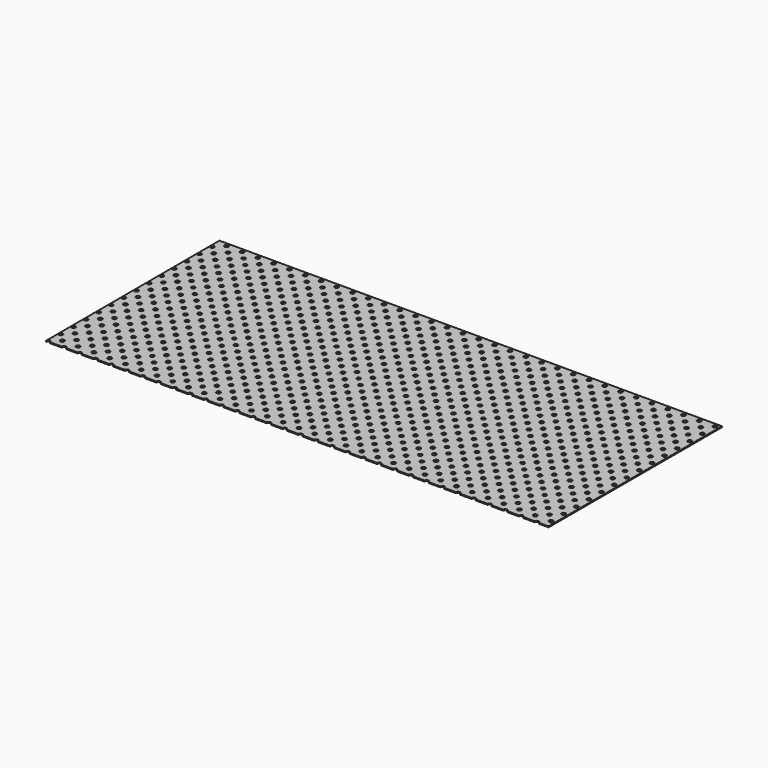
from build123d import *

# Parameters (mm, degrees)
F0_R     = 2
F1_DEPTH = 1


with BuildPart() as f1:
    # F0 (on Top) → F1 (new body)
    with BuildSketch(Plane.XY):
        with BuildLine():
            Line((245.0974984355, -110), (255, -110))
            Line((255, -110), (255, 110))
            Line((255, 110), (-255, 110))
            Line((-255, 110), (-255, -110))
            Line((-255, -110), (-254.8974984355, -110))
            ThreePointArc((-254.8974984355, -110), (-252.9500156421, -107.9006254889), (-250.9, -109.9))
            ThreePointArc((-250.9, -109.9), (-250.9006254889, -109.9500156421), (-250.9025015645, -110))
            Line((-250.9025015645, -110), (-238.8974984355, -110))
            ThreePointArc((-238.8974984355, -110), (-236.9500156421, -107.9006254889), (-234.9, -109.9))
            ThreePointArc((-234.9, -109.9), (-234.9006254889, -109.9500156421), (-234.9025015645, -110))
            Line((-234.9025015645, -110), (-222.8974984355, -110))
            ThreePointArc((-222.8974984355, -110), (-220.9500156421, -107.9006254889), (-218.9, -109.9))
            ThreePointArc((-218.9, -109.9), (-218.9006254889, -109.9500156421), (-218.9025015645, -110))
            Line((-218.9025015645, -110), (-206.8974984355, -110))
            ThreePointArc((-206.8974984355, -110), (-204.9500156421, -107.9006254889), (-202.9, -109.9))
            ThreePointArc((-202.9, -109.9), (-202.9006254889, -109.9500156421), (-202.9025015645, -110))
            Line((-202.9025015645, -110), (-190.8974984355, -110))
            ThreePointArc((-190.8974984355, -110), (-188.9500156421, -107.9006254889), (-186.9, -109.9))
            ThreePointArc((-186.9, -109.9), (-186.9006254889, -109.9500156421), (-186.9025015645, -110))
            Line((-186.9025015645, -110), (-174.8974984355, -110))
            ThreePointArc((-174.8974984355, -110), (-172.9500156421, -107.9006254889), (-170.9, -109.9))
            ThreePointArc((-170.9, -109.9), (-170.9006254889, -109.9500156421), (-170.9025015645, -110))
            Line((-170.9025015645, -110), (-158.8974984355, -110))
            ThreePointArc((-158.8974984355, -110), (-156.9500156421, -107.9006254889), (-154.9, -109.9))
            ThreePointArc((-154.9, -109.9), (-154.9006254889, -109.9500156421), (-154.9025015645, -110))
            Line((-154.9025015645, -110), (-142.8974984355, -110))
            ThreePointArc((-142.8974984355, -110), (-140.9500156421, -107.9006254889), (-138.9, -109.9))
            ThreePointArc((-138.9, -109.9), (-138.9006254889, -109.9500156421), (-138.9025015645, -110))
            Line((-138.9025015645, -110), (-126.8974984355, -110))
            ThreePointArc((-126.8974984355, -110), (-124.9500156421, -107.9006254889), (-122.9, -109.9))
            ThreePointArc((-122.9, -109.9), (-122.9006254889, -109.9500156421), (-122.9025015645, -110))
            Line((-122.9025015645, -110), (-110.8974984355, -110))
            ThreePointArc((-110.8974984355, -110), (-108.9500156421, -107.9006254889), (-106.9, -109.9))
            ThreePointArc((-106.9, -109.9), (-106.9006254889, -109.9500156421), (-106.9025015645, -110))
            Line((-106.9025015645, -110), (-94.8974984355, -110))
            ThreePointArc((-94.8974984355, -110), (-92.9500156421, -107.9006254889), (-90.9, -109.9))
            ThreePointArc((-90.9, -109.9), (-90.9006254889, -109.9500156421), (-90.9025015645, -110))
            Line((-90.9025015645, -110), (-78.8974984355, -110))
            ThreePointArc((-78.8974984355, -110), (-76.9500156421, -107.9006254889), (-74.9, -109.9))
            ThreePointArc((-74.9, -109.9), (-74.9006254889, -109.9500156421), (-74.9025015645, -110))
            Line((-74.9025015645, -110), (-62.8974984355, -110))
            ThreePointArc((-62.8974984355, -110), (-60.9500156421, -107.9006254889), (-58.9, -109.9))
            ThreePointArc((-58.9, -109.9), (-58.9006254889, -109.9500156421), (-58.9025015645, -110))
            Line((-58.9025015645, -110), (-46.8974984355, -110))
            ThreePointArc((-46.8974984355, -110), (-44.9500156421, -107.9006254889), (-42.9, -109.9))
            ThreePointArc((-42.9, -109.9), (-42.9006254889, -109.9500156421), (-42.9025015645, -110))
            Line((-42.9025015645, -110), (-30.8974984355, -110))
            ThreePointArc((-30.8974984355, -110), (-28.9500156421, -107.9006254889), (-26.9, -109.9))
            ThreePointArc((-26.9, -109.9), (-26.9006254889, -109.9500156421), (-26.9025015645, -110))
            Line((-26.9025015645, -110), (-14.8974984355, -110))
            ThreePointArc((-14.8974984355, -110), (-12.9500156421, -107.9006254889), (-10.9, -109.9))
            ThreePointArc((-10.9, -109.9), (-10.9006254889, -109.9500156421), (-10.9025015645, -110))
            Line((-10.9025015645, -110), (1.1025015645, -110))
            ThreePointArc((1.1025015645, -110), (3.0499843579, -107.9006254889), (5.1, -109.9))
            ThreePointArc((5.1, -109.9), (5.0993745111, -109.9500156421), (5.0974984355, -110))
            Line((5.0974984355, -110), (17.1025015645, -110))
            ThreePointArc((17.1025015645, -110), (19.0499843579, -107.9006254889), (21.1, -109.9))
            ThreePointArc((21.1, -109.9), (21.0993745111, -109.9500156421), (21.0974984355, -110))
            Line((21.0974984355, -110), (33.1025015645, -110))
            ThreePointArc((33.1025015645, -110), (35.0499843579, -107.9006254889), (37.1, -109.9))
            ThreePointArc((37.1, -109.9), (37.0993745111, -109.9500156421), (37.0974984355, -110))
            Line((37.0974984355, -110), (49.1025015645, -110))
            ThreePointArc((49.1025015645, -110), (51.0499843579, -107.9006254889), (53.1, -109.9))
            ThreePointArc((53.1, -109.9), (53.0993745111, -109.9500156421), (53.0974984355, -110))
            Line((53.0974984355, -110), (65.1025015645, -110))
            ThreePointArc((65.1025015645, -110), (67.0499843579, -107.9006254889), (69.1, -109.9))
            ThreePointArc((69.1, -109.9), (69.0993745111, -109.9500156421), (69.0974984355, -110))
            Line((69.0974984355, -110), (81.1025015645, -110))
            ThreePointArc((81.1025015645, -110), (83.0499843579, -107.9006254889), (85.1, -109.9))
            ThreePointArc((85.1, -109.9), (85.0993745111, -109.9500156421), (85.0974984355, -110))
            Line((85.0974984355, -110), (97.1025015645, -110))
            ThreePointArc((97.1025015645, -110), (99.0499843579, -107.9006254889), (101.1, -109.9))
            ThreePointArc((101.1, -109.9), (101.0993745111, -109.9500156421), (101.0974984355, -110))
            Line((101.0974984355, -110), (113.1025015645, -110))
            ThreePointArc((113.1025015645, -110), (115.0499843579, -107.9006254889), (117.1, -109.9))
            ThreePointArc((117.1, -109.9), (117.0993745111, -109.9500156421), (117.0974984355, -110))
            Line((117.0974984355, -110), (129.1025015645, -110))
            ThreePointArc((129.1025015645, -110), (131.0499843579, -107.9006254889), (133.1, -109.9))
            ThreePointArc((133.1, -109.9), (133.0993745111, -109.9500156421), (133.0974984355, -110))
            Line((133.0974984355, -110), (145.1025015645, -110))
            ThreePointArc((145.1025015645, -110), (147.0499843579, -107.9006254889), (149.1, -109.9))
            ThreePointArc((149.1, -109.9), (149.0993745111, -109.9500156421), (149.0974984355, -110))
            Line((149.0974984355, -110), (161.1025015645, -110))
            ThreePointArc((161.1025015645, -110), (163.0499843579, -107.9006254889), (165.1, -109.9))
            ThreePointArc((165.1, -109.9), (165.0993745111, -109.9500156421), (165.0974984355, -110))
            Line((165.0974984355, -110), (177.1025015645, -110))
            ThreePointArc((177.1025015645, -110), (179.0499843579, -107.9006254889), (181.1, -109.9))
            ThreePointArc((181.1, -109.9), (181.0993745111, -109.9500156421), (181.0974984355, -110))
            Line((181.0974984355, -110), (193.1025015645, -110))
            ThreePointArc((193.1025015645, -110), (195.0499843579, -107.9006254889), (197.1, -109.9))
            ThreePointArc((197.1, -109.9), (197.0993745111, -109.9500156421), (197.0974984355, -110))
            Line((197.0974984355, -110), (209.1025015645, -110))
            ThreePointArc((209.1025015645, -110), (211.0499843579, -107.9006254889), (213.1, -109.9))
            ThreePointArc((213.1, -109.9), (213.0993745111, -109.9500156421), (213.0974984355, -110))
            Line((213.0974984355, -110), (225.1025015645, -110))
            ThreePointArc((225.1025015645, -110), (227.0499843579, -107.9006254889), (229.1, -109.9))
            ThreePointArc((229.1, -109.9), (229.0993745111, -109.9500156421), (229.0974984355, -110))
            Line((229.0974984355, -110), (241.1025015645, -110))
            ThreePointArc((241.1025015645, -110), (243.0499843579, -107.9006254889), (245.1, -109.9))
            ThreePointArc((245.1, -109.9), (245.0993745111, -109.9500156421), (245.0974984355, -110))
        make_face()
        with Locations((-244.9, -101.9)):
            Circle(F0_R, mode=Mode.SUBTRACT)
        with Locations((-228.9, -101.9)):
            Circle(F0_R, mode=Mode.SUBTRACT)
        with Locations((-212.9, -101.9)):
            Circle(F0_R, mode=Mode.SUBTRACT)
        with Locations((-196.9, -101.9)):
            Circle(F0_R, mode=Mode.SUBTRACT)
        with Locations((-252.9, -93.9)):
            Circle(F0_R, mode=Mode.SUBTRACT)
        with Locations((-236.9, -93.9)):
            Circle(F0_R, mode=Mode.SUBTRACT)
        with Locations((-244.9, -85.9)):
            Circle(F0_R, mode=Mode.SUBTRACT)
        with Locations((-228.9, -85.9)):
            Circle(F0_R, mode=Mode.SUBTRACT)
        with Locations((-220.9, -93.9)):
            Circle(F0_R, mode=Mode.SUBTRACT)
        with Locations((-204.9, -93.9)):
            Circle(F0_R, mode=Mode.SUBTRACT)
        with Locations((-212.9, -85.9)):
            Circle(F0_R, mode=Mode.SUBTRACT)
        with Locations((-196.9, -85.9)):
            Circle(F0_R, mode=Mode.SUBTRACT)
        with Locations((-180.9, -101.9)):
            Circle(F0_R, mode=Mode.SUBTRACT)
        with Locations((-164.9, -101.9)):
            Circle(F0_R, mode=Mode.SUBTRACT)
        with Locations((-148.9, -101.9)):
            Circle(F0_R, mode=Mode.SUBTRACT)
        with Locations((-132.9, -101.9)):
            Circle(F0_R, mode=Mode.SUBTRACT)
        with Locations((-188.9, -93.9)):
            Circle(F0_R, mode=Mode.SUBTRACT)
        with Locations((-172.9, -93.9)):
            Circle(F0_R, mode=Mode.SUBTRACT)
        with Locations((-156.9, -93.9)):
            Circle(F0_R, mode=Mode.SUBTRACT)
        with Locations((-180.9, -85.9)):
            Circle(F0_R, mode=Mode.SUBTRACT)
        with Locations((-164.9, -85.9)):
            Circle(F0_R, mode=Mode.SUBTRACT)
        with Locations((-140.9, -93.9)):
            Circle(F0_R, mode=Mode.SUBTRACT)
        with Locations((-124.9, -93.9)):
            Circle(F0_R, mode=Mode.SUBTRACT)
        with Locations((-148.9, -85.9)):
            Circle(F0_R, mode=Mode.SUBTRACT)
        with Locations((-132.9, -85.9)):
            Circle(F0_R, mode=Mode.SUBTRACT)
        with Locations((-252.9, -77.9)):
            Circle(F0_R, mode=Mode.SUBTRACT)
        with Locations((-236.9, -77.9)):
            Circle(F0_R, mode=Mode.SUBTRACT)
        with Locations((-220.9, -77.9)):
            Circle(F0_R, mode=Mode.SUBTRACT)
        with Locations((-204.9, -77.9)):
            Circle(F0_R, mode=Mode.SUBTRACT)
        with Locations((-244.9, -69.9)):
            Circle(F0_R, mode=Mode.SUBTRACT)
        with Locations((-228.9, -69.9)):
            Circle(F0_R, mode=Mode.SUBTRACT)
        with Locations((-252.9, -61.9)):
            Circle(F0_R, mode=Mode.SUBTRACT)
        with Locations((-236.9, -61.9)):
            Circle(F0_R, mode=Mode.SUBTRACT)
        with Locations((-212.9, -69.9)):
            Circle(F0_R, mode=Mode.SUBTRACT)
        with Locations((-196.9, -69.9)):
            Circle(F0_R, mode=Mode.SUBTRACT)
        with Locations((-220.9, -61.9)):
            Circle(F0_R, mode=Mode.SUBTRACT)
        with Locations((-204.9, -61.9)):
            Circle(F0_R, mode=Mode.SUBTRACT)
        with Locations((-188.9, -77.9)):
            Circle(F0_R, mode=Mode.SUBTRACT)
        with Locations((-172.9, -77.9)):
            Circle(F0_R, mode=Mode.SUBTRACT)
        with Locations((-156.9, -77.9)):
            Circle(F0_R, mode=Mode.SUBTRACT)
        with Locations((-140.9, -77.9)):
            Circle(F0_R, mode=Mode.SUBTRACT)
        with Locations((-124.9, -77.9)):
            Circle(F0_R, mode=Mode.SUBTRACT)
        with Locations((-180.9, -69.9)):
            Circle(F0_R, mode=Mode.SUBTRACT)
        with Locations((-164.9, -69.9)):
            Circle(F0_R, mode=Mode.SUBTRACT)
        with Locations((-188.9, -61.9)):
            Circle(F0_R, mode=Mode.SUBTRACT)
        with Locations((-172.9, -61.9)):
            Circle(F0_R, mode=Mode.SUBTRACT)
        with Locations((-156.9, -61.9)):
            Circle(F0_R, mode=Mode.SUBTRACT)
        with Locations((-148.9, -69.9)):
            Circle(F0_R, mode=Mode.SUBTRACT)
        with Locations((-132.9, -69.9)):
            Circle(F0_R, mode=Mode.SUBTRACT)
        with Locations((-140.9, -61.9)):
            Circle(F0_R, mode=Mode.SUBTRACT)
        with Locations((-124.9, -61.9)):
            Circle(F0_R, mode=Mode.SUBTRACT)
        with Locations((-116.9, -101.9)):
            Circle(F0_R, mode=Mode.SUBTRACT)
        with Locations((-100.9, -101.9)):
            Circle(F0_R, mode=Mode.SUBTRACT)
        with Locations((-84.9, -101.9)):
            Circle(F0_R, mode=Mode.SUBTRACT)
        with Locations((-68.9, -101.9)):
            Circle(F0_R, mode=Mode.SUBTRACT)
        with Locations((-108.9, -93.9)):
            Circle(F0_R, mode=Mode.SUBTRACT)
        with Locations((-92.9, -93.9)):
            Circle(F0_R, mode=Mode.SUBTRACT)
        with Locations((-116.9, -85.9)):
            Circle(F0_R, mode=Mode.SUBTRACT)
        with Locations((-100.9, -85.9)):
            Circle(F0_R, mode=Mode.SUBTRACT)
        with Locations((-76.9, -93.9)):
            Circle(F0_R, mode=Mode.SUBTRACT)
        with Locations((-60.9, -93.9)):
            Circle(F0_R, mode=Mode.SUBTRACT)
        with Locations((-84.9, -85.9)):
            Circle(F0_R, mode=Mode.SUBTRACT)
        with Locations((-68.9, -85.9)):
            Circle(F0_R, mode=Mode.SUBTRACT)
        with Locations((-52.9, -101.9)):
            Circle(F0_R, mode=Mode.SUBTRACT)
        with Locations((-36.9, -101.9)):
            Circle(F0_R, mode=Mode.SUBTRACT)
        with Locations((-20.9, -101.9)):
            Circle(F0_R, mode=Mode.SUBTRACT)
        with Locations((-4.9, -101.9)):
            Circle(F0_R, mode=Mode.SUBTRACT)
        with Locations((-44.9, -93.9)):
            Circle(F0_R, mode=Mode.SUBTRACT)
        with Locations((-28.9, -93.9)):
            Circle(F0_R, mode=Mode.SUBTRACT)
        with Locations((-52.9, -85.9)):
            Circle(F0_R, mode=Mode.SUBTRACT)
        with Locations((-36.9, -85.9)):
            Circle(F0_R, mode=Mode.SUBTRACT)
        with Locations((-12.9, -93.9)):
            Circle(F0_R, mode=Mode.SUBTRACT)
        with Locations((3.1, -93.9)):
            Circle(F0_R, mode=Mode.SUBTRACT)
        with Locations((-20.9, -85.9)):
            Circle(F0_R, mode=Mode.SUBTRACT)
        with Locations((-4.9, -85.9)):
            Circle(F0_R, mode=Mode.SUBTRACT)
        with Locations((-108.9, -77.9)):
            Circle(F0_R, mode=Mode.SUBTRACT)
        with Locations((-92.9, -77.9)):
            Circle(F0_R, mode=Mode.SUBTRACT)
        with Locations((-76.9, -77.9)):
            Circle(F0_R, mode=Mode.SUBTRACT)
        with Locations((-60.9, -77.9)):
            Circle(F0_R, mode=Mode.SUBTRACT)
        with Locations((-116.9, -69.9)):
            Circle(F0_R, mode=Mode.SUBTRACT)
        with Locations((-100.9, -69.9)):
            Circle(F0_R, mode=Mode.SUBTRACT)
        with Locations((-108.9, -61.9)):
            Circle(F0_R, mode=Mode.SUBTRACT)
        with Locations((-92.9, -61.9)):
            Circle(F0_R, mode=Mode.SUBTRACT)
        with Locations((-84.9, -69.9)):
            Circle(F0_R, mode=Mode.SUBTRACT)
        with Locations((-68.9, -69.9)):
            Circle(F0_R, mode=Mode.SUBTRACT)
        with Locations((-76.9, -61.9)):
            Circle(F0_R, mode=Mode.SUBTRACT)
        with Locations((-60.9, -61.9)):
            Circle(F0_R, mode=Mode.SUBTRACT)
        with Locations((-44.9, -77.9)):
            Circle(F0_R, mode=Mode.SUBTRACT)
        with Locations((-28.9, -77.9)):
            Circle(F0_R, mode=Mode.SUBTRACT)
        with Locations((-12.9, -77.9)):
            Circle(F0_R, mode=Mode.SUBTRACT)
        with Locations((3.1, -77.9)):
            Circle(F0_R, mode=Mode.SUBTRACT)
        with Locations((-52.9, -69.9)):
            Circle(F0_R, mode=Mode.SUBTRACT)
        with Locations((-36.9, -69.9)):
            Circle(F0_R, mode=Mode.SUBTRACT)
        with Locations((-44.9, -61.9)):
            Circle(F0_R, mode=Mode.SUBTRACT)
        with Locations((-28.9, -61.9)):
            Circle(F0_R, mode=Mode.SUBTRACT)
        with Locations((-20.9, -69.9)):
            Circle(F0_R, mode=Mode.SUBTRACT)
        with Locations((-4.9, -69.9)):
            Circle(F0_R, mode=Mode.SUBTRACT)
        with Locations((-12.9, -61.9)):
            Circle(F0_R, mode=Mode.SUBTRACT)
        with Locations((3.1, -61.9)):
            Circle(F0_R, mode=Mode.SUBTRACT)
        with Locations((-244.9, -53.9)):
            Circle(F0_R, mode=Mode.SUBTRACT)
        with Locations((-228.9, -53.9)):
            Circle(F0_R, mode=Mode.SUBTRACT)
        with Locations((-252.9, -45.9)):
            Circle(F0_R, mode=Mode.SUBTRACT)
        with Locations((-236.9, -45.9)):
            Circle(F0_R, mode=Mode.SUBTRACT)
        with Locations((-212.9, -53.9)):
            Circle(F0_R, mode=Mode.SUBTRACT)
        with Locations((-196.9, -53.9)):
            Circle(F0_R, mode=Mode.SUBTRACT)
        with Locations((-220.9, -45.9)):
            Circle(F0_R, mode=Mode.SUBTRACT)
        with Locations((-204.9, -45.9)):
            Circle(F0_R, mode=Mode.SUBTRACT)
        with Locations((-244.9, -37.9)):
            Circle(F0_R, mode=Mode.SUBTRACT)
        with Locations((-228.9, -37.9)):
            Circle(F0_R, mode=Mode.SUBTRACT)
        with Locations((-252.9, -29.9)):
            Circle(F0_R, mode=Mode.SUBTRACT)
        with Locations((-236.9, -29.9)):
            Circle(F0_R, mode=Mode.SUBTRACT)
        with Locations((-212.9, -37.9)):
            Circle(F0_R, mode=Mode.SUBTRACT)
        with Locations((-196.9, -37.9)):
            Circle(F0_R, mode=Mode.SUBTRACT)
        with Locations((-220.9, -29.9)):
            Circle(F0_R, mode=Mode.SUBTRACT)
        with Locations((-204.9, -29.9)):
            Circle(F0_R, mode=Mode.SUBTRACT)
        with Locations((-180.9, -53.9)):
            Circle(F0_R, mode=Mode.SUBTRACT)
        with Locations((-164.9, -53.9)):
            Circle(F0_R, mode=Mode.SUBTRACT)
        with Locations((-188.9, -45.9)):
            Circle(F0_R, mode=Mode.SUBTRACT)
        with Locations((-172.9, -45.9)):
            Circle(F0_R, mode=Mode.SUBTRACT)
        with Locations((-156.9, -45.9)):
            Circle(F0_R, mode=Mode.SUBTRACT)
        with Locations((-148.9, -53.9)):
            Circle(F0_R, mode=Mode.SUBTRACT)
        with Locations((-132.9, -53.9)):
            Circle(F0_R, mode=Mode.SUBTRACT)
        with Locations((-140.9, -45.9)):
            Circle(F0_R, mode=Mode.SUBTRACT)
        with Locations((-124.9, -45.9)):
            Circle(F0_R, mode=Mode.SUBTRACT)
        with Locations((-180.9, -37.9)):
            Circle(F0_R, mode=Mode.SUBTRACT)
        with Locations((-164.9, -37.9)):
            Circle(F0_R, mode=Mode.SUBTRACT)
        with Locations((-188.9, -29.9)):
            Circle(F0_R, mode=Mode.SUBTRACT)
        with Locations((-172.9, -29.9)):
            Circle(F0_R, mode=Mode.SUBTRACT)
        with Locations((-156.9, -29.9)):
            Circle(F0_R, mode=Mode.SUBTRACT)
        with Locations((-148.9, -37.9)):
            Circle(F0_R, mode=Mode.SUBTRACT)
        with Locations((-132.9, -37.9)):
            Circle(F0_R, mode=Mode.SUBTRACT)
        with Locations((-140.9, -29.9)):
            Circle(F0_R, mode=Mode.SUBTRACT)
        with Locations((-124.9, -29.9)):
            Circle(F0_R, mode=Mode.SUBTRACT)
        with Locations((-244.9, -21.9)):
            Circle(F0_R, mode=Mode.SUBTRACT)
        with Locations((-228.9, -21.9)):
            Circle(F0_R, mode=Mode.SUBTRACT)
        with Locations((-212.9, -21.9)):
            Circle(F0_R, mode=Mode.SUBTRACT)
        with Locations((-196.9, -21.9)):
            Circle(F0_R, mode=Mode.SUBTRACT)
        with Locations((-252.9, -13.9)):
            Circle(F0_R, mode=Mode.SUBTRACT)
        with Locations((-236.9, -13.9)):
            Circle(F0_R, mode=Mode.SUBTRACT)
        with Locations((-244.9, -5.9)):
            Circle(F0_R, mode=Mode.SUBTRACT)
        with Locations((-228.9, -5.9)):
            Circle(F0_R, mode=Mode.SUBTRACT)
        with Locations((-220.9, -13.9)):
            Circle(F0_R, mode=Mode.SUBTRACT)
        with Locations((-204.9, -13.9)):
            Circle(F0_R, mode=Mode.SUBTRACT)
        with Locations((-212.9, -5.9)):
            Circle(F0_R, mode=Mode.SUBTRACT)
        with Locations((-196.9, -5.9)):
            Circle(F0_R, mode=Mode.SUBTRACT)
        with Locations((-180.9, -21.9)):
            Circle(F0_R, mode=Mode.SUBTRACT)
        with Locations((-164.9, -21.9)):
            Circle(F0_R, mode=Mode.SUBTRACT)
        with Locations((-148.9, -21.9)):
            Circle(F0_R, mode=Mode.SUBTRACT)
        with Locations((-132.9, -21.9)):
            Circle(F0_R, mode=Mode.SUBTRACT)
        with Locations((-188.9, -13.9)):
            Circle(F0_R, mode=Mode.SUBTRACT)
        with Locations((-172.9, -13.9)):
            Circle(F0_R, mode=Mode.SUBTRACT)
        with Locations((-156.9, -13.9)):
            Circle(F0_R, mode=Mode.SUBTRACT)
        with Locations((-180.9, -5.9)):
            Circle(F0_R, mode=Mode.SUBTRACT)
        with Locations((-164.9, -5.9)):
            Circle(F0_R, mode=Mode.SUBTRACT)
        with Locations((-140.9, -13.9)):
            Circle(F0_R, mode=Mode.SUBTRACT)
        with Locations((-124.9, -13.9)):
            Circle(F0_R, mode=Mode.SUBTRACT)
        with Locations((-148.9, -5.9)):
            Circle(F0_R, mode=Mode.SUBTRACT)
        with Locations((-132.9, -5.9)):
            Circle(F0_R, mode=Mode.SUBTRACT)
        with Locations((-116.9, -53.9)):
            Circle(F0_R, mode=Mode.SUBTRACT)
        with Locations((-100.9, -53.9)):
            Circle(F0_R, mode=Mode.SUBTRACT)
        with Locations((-108.9, -45.9)):
            Circle(F0_R, mode=Mode.SUBTRACT)
        with Locations((-92.9, -45.9)):
            Circle(F0_R, mode=Mode.SUBTRACT)
        with Locations((-84.9, -53.9)):
            Circle(F0_R, mode=Mode.SUBTRACT)
        with Locations((-68.9, -53.9)):
            Circle(F0_R, mode=Mode.SUBTRACT)
        with Locations((-76.9, -45.9)):
            Circle(F0_R, mode=Mode.SUBTRACT)
        with Locations((-60.9, -45.9)):
            Circle(F0_R, mode=Mode.SUBTRACT)
        with Locations((-116.9, -37.9)):
            Circle(F0_R, mode=Mode.SUBTRACT)
        with Locations((-100.9, -37.9)):
            Circle(F0_R, mode=Mode.SUBTRACT)
        with Locations((-108.9, -29.9)):
            Circle(F0_R, mode=Mode.SUBTRACT)
        with Locations((-92.9, -29.9)):
            Circle(F0_R, mode=Mode.SUBTRACT)
        with Locations((-84.9, -37.9)):
            Circle(F0_R, mode=Mode.SUBTRACT)
        with Locations((-68.9, -37.9)):
            Circle(F0_R, mode=Mode.SUBTRACT)
        with Locations((-76.9, -29.9)):
            Circle(F0_R, mode=Mode.SUBTRACT)
        with Locations((-60.9, -29.9)):
            Circle(F0_R, mode=Mode.SUBTRACT)
        with Locations((-52.9, -53.9)):
            Circle(F0_R, mode=Mode.SUBTRACT)
        with Locations((-36.9, -53.9)):
            Circle(F0_R, mode=Mode.SUBTRACT)
        with Locations((-44.9, -45.9)):
            Circle(F0_R, mode=Mode.SUBTRACT)
        with Locations((-28.9, -45.9)):
            Circle(F0_R, mode=Mode.SUBTRACT)
        with Locations((-20.9, -53.9)):
            Circle(F0_R, mode=Mode.SUBTRACT)
        with Locations((-4.9, -53.9)):
            Circle(F0_R, mode=Mode.SUBTRACT)
        with Locations((-12.9, -45.9)):
            Circle(F0_R, mode=Mode.SUBTRACT)
        with Locations((3.1, -45.9)):
            Circle(F0_R, mode=Mode.SUBTRACT)
        with Locations((-52.9, -37.9)):
            Circle(F0_R, mode=Mode.SUBTRACT)
        with Locations((-36.9, -37.9)):
            Circle(F0_R, mode=Mode.SUBTRACT)
        with Locations((-44.9, -29.9)):
            Circle(F0_R, mode=Mode.SUBTRACT)
        with Locations((-28.9, -29.9)):
            Circle(F0_R, mode=Mode.SUBTRACT)
        with Locations((-20.9, -37.9)):
            Circle(F0_R, mode=Mode.SUBTRACT)
        with Locations((-4.9, -37.9)):
            Circle(F0_R, mode=Mode.SUBTRACT)
        with Locations((-12.9, -29.9)):
            Circle(F0_R, mode=Mode.SUBTRACT)
        with Locations((3.1, -29.9)):
            Circle(F0_R, mode=Mode.SUBTRACT)
        with Locations((-116.9, -21.9)):
            Circle(F0_R, mode=Mode.SUBTRACT)
        with Locations((-100.9, -21.9)):
            Circle(F0_R, mode=Mode.SUBTRACT)
        with Locations((-84.9, -21.9)):
            Circle(F0_R, mode=Mode.SUBTRACT)
        with Locations((-68.9, -21.9)):
            Circle(F0_R, mode=Mode.SUBTRACT)
        with Locations((-108.9, -13.9)):
            Circle(F0_R, mode=Mode.SUBTRACT)
        with Locations((-92.9, -13.9)):
            Circle(F0_R, mode=Mode.SUBTRACT)
        with Locations((-116.9, -5.9)):
            Circle(F0_R, mode=Mode.SUBTRACT)
        with Locations((-100.9, -5.9)):
            Circle(F0_R, mode=Mode.SUBTRACT)
        with Locations((-76.9, -13.9)):
            Circle(F0_R, mode=Mode.SUBTRACT)
        with Locations((-60.9, -13.9)):
            Circle(F0_R, mode=Mode.SUBTRACT)
        with Locations((-84.9, -5.9)):
            Circle(F0_R, mode=Mode.SUBTRACT)
        with Locations((-68.9, -5.9)):
            Circle(F0_R, mode=Mode.SUBTRACT)
        with Locations((-52.9, -21.9)):
            Circle(F0_R, mode=Mode.SUBTRACT)
        with Locations((-36.9, -21.9)):
            Circle(F0_R, mode=Mode.SUBTRACT)
        with Locations((-20.9, -21.9)):
            Circle(F0_R, mode=Mode.SUBTRACT)
        with Locations((-4.9, -21.9)):
            Circle(F0_R, mode=Mode.SUBTRACT)
        with Locations((-44.9, -13.9)):
            Circle(F0_R, mode=Mode.SUBTRACT)
        with Locations((-28.9, -13.9)):
            Circle(F0_R, mode=Mode.SUBTRACT)
        with Locations((-52.9, -5.9)):
            Circle(F0_R, mode=Mode.SUBTRACT)
        with Locations((-36.9, -5.9)):
            Circle(F0_R, mode=Mode.SUBTRACT)
        with Locations((-12.9, -13.9)):
            Circle(F0_R, mode=Mode.SUBTRACT)
        with Locations((3.1, -13.9)):
            Circle(F0_R, mode=Mode.SUBTRACT)
        with Locations((-20.9, -5.9)):
            Circle(F0_R, mode=Mode.SUBTRACT)
        with Locations((-4.9, -5.9)):
            Circle(F0_R, mode=Mode.SUBTRACT)
        with Locations((11.1, -101.9)):
            Circle(F0_R, mode=Mode.SUBTRACT)
        with Locations((27.1, -101.9)):
            Circle(F0_R, mode=Mode.SUBTRACT)
        with Locations((43.1, -101.9)):
            Circle(F0_R, mode=Mode.SUBTRACT)
        with Locations((59.1, -101.9)):
            Circle(F0_R, mode=Mode.SUBTRACT)
        with Locations((19.1, -93.9)):
            Circle(F0_R, mode=Mode.SUBTRACT)
        with Locations((35.1, -93.9)):
            Circle(F0_R, mode=Mode.SUBTRACT)
        with Locations((11.1, -85.9)):
            Circle(F0_R, mode=Mode.SUBTRACT)
        with Locations((27.1, -85.9)):
            Circle(F0_R, mode=Mode.SUBTRACT)
        with Locations((51.1, -93.9)):
            Circle(F0_R, mode=Mode.SUBTRACT)
        with Locations((67.1, -93.9)):
            Circle(F0_R, mode=Mode.SUBTRACT)
        with Locations((43.1, -85.9)):
            Circle(F0_R, mode=Mode.SUBTRACT)
        with Locations((59.1, -85.9)):
            Circle(F0_R, mode=Mode.SUBTRACT)
        with Locations((75.1, -101.9)):
            Circle(F0_R, mode=Mode.SUBTRACT)
        with Locations((91.1, -101.9)):
            Circle(F0_R, mode=Mode.SUBTRACT)
        with Locations((107.1, -101.9)):
            Circle(F0_R, mode=Mode.SUBTRACT)
        with Locations((123.1, -101.9)):
            Circle(F0_R, mode=Mode.SUBTRACT)
        with Locations((83.1, -93.9)):
            Circle(F0_R, mode=Mode.SUBTRACT)
        with Locations((99.1, -93.9)):
            Circle(F0_R, mode=Mode.SUBTRACT)
        with Locations((75.1, -85.9)):
            Circle(F0_R, mode=Mode.SUBTRACT)
        with Locations((91.1, -85.9)):
            Circle(F0_R, mode=Mode.SUBTRACT)
        with Locations((115.1, -93.9)):
            Circle(F0_R, mode=Mode.SUBTRACT)
        with Locations((131.1, -93.9)):
            Circle(F0_R, mode=Mode.SUBTRACT)
        with Locations((107.1, -85.9)):
            Circle(F0_R, mode=Mode.SUBTRACT)
        with Locations((123.1, -85.9)):
            Circle(F0_R, mode=Mode.SUBTRACT)
        with Locations((19.1, -77.9)):
            Circle(F0_R, mode=Mode.SUBTRACT)
        with Locations((35.1, -77.9)):
            Circle(F0_R, mode=Mode.SUBTRACT)
        with Locations((51.1, -77.9)):
            Circle(F0_R, mode=Mode.SUBTRACT)
        with Locations((67.1, -77.9)):
            Circle(F0_R, mode=Mode.SUBTRACT)
        with Locations((11.1, -69.9)):
            Circle(F0_R, mode=Mode.SUBTRACT)
        with Locations((27.1, -69.9)):
            Circle(F0_R, mode=Mode.SUBTRACT)
        with Locations((19.1, -61.9)):
            Circle(F0_R, mode=Mode.SUBTRACT)
        with Locations((35.1, -61.9)):
            Circle(F0_R, mode=Mode.SUBTRACT)
        with Locations((43.1, -69.9)):
            Circle(F0_R, mode=Mode.SUBTRACT)
        with Locations((59.1, -69.9)):
            Circle(F0_R, mode=Mode.SUBTRACT)
        with Locations((51.1, -61.9)):
            Circle(F0_R, mode=Mode.SUBTRACT)
        with Locations((67.1, -61.9)):
            Circle(F0_R, mode=Mode.SUBTRACT)
        with Locations((83.1, -77.9)):
            Circle(F0_R, mode=Mode.SUBTRACT)
        with Locations((99.1, -77.9)):
            Circle(F0_R, mode=Mode.SUBTRACT)
        with Locations((115.1, -77.9)):
            Circle(F0_R, mode=Mode.SUBTRACT)
        with Locations((131.1, -77.9)):
            Circle(F0_R, mode=Mode.SUBTRACT)
        with Locations((75.1, -69.9)):
            Circle(F0_R, mode=Mode.SUBTRACT)
        with Locations((91.1, -69.9)):
            Circle(F0_R, mode=Mode.SUBTRACT)
        with Locations((83.1, -61.9)):
            Circle(F0_R, mode=Mode.SUBTRACT)
        with Locations((99.1, -61.9)):
            Circle(F0_R, mode=Mode.SUBTRACT)
        with Locations((107.1, -69.9)):
            Circle(F0_R, mode=Mode.SUBTRACT)
        with Locations((123.1, -69.9)):
            Circle(F0_R, mode=Mode.SUBTRACT)
        with Locations((115.1, -61.9)):
            Circle(F0_R, mode=Mode.SUBTRACT)
        with Locations((131.1, -61.9)):
            Circle(F0_R, mode=Mode.SUBTRACT)
        with Locations((139.1, -101.9)):
            Circle(F0_R, mode=Mode.SUBTRACT)
        with Locations((155.1, -101.9)):
            Circle(F0_R, mode=Mode.SUBTRACT)
        with Locations((171.1, -101.9)):
            Circle(F0_R, mode=Mode.SUBTRACT)
        with Locations((187.1, -101.9)):
            Circle(F0_R, mode=Mode.SUBTRACT)
        with Locations((203.1, -101.9)):
            Circle(F0_R, mode=Mode.SUBTRACT)
        with Locations((147.1, -93.9)):
            Circle(F0_R, mode=Mode.SUBTRACT)
        with Locations((163.1, -93.9)):
            Circle(F0_R, mode=Mode.SUBTRACT)
        with Locations((139.1, -85.9)):
            Circle(F0_R, mode=Mode.SUBTRACT)
        with Locations((155.1, -85.9)):
            Circle(F0_R, mode=Mode.SUBTRACT)
        with Locations((179.1, -93.9)):
            Circle(F0_R, mode=Mode.SUBTRACT)
        with Locations((195.1, -93.9)):
            Circle(F0_R, mode=Mode.SUBTRACT)
        with Locations((171.1, -85.9)):
            Circle(F0_R, mode=Mode.SUBTRACT)
        with Locations((187.1, -85.9)):
            Circle(F0_R, mode=Mode.SUBTRACT)
        with Locations((203.1, -85.9)):
            Circle(F0_R, mode=Mode.SUBTRACT)
        with Locations((219.1, -101.9)):
            Circle(F0_R, mode=Mode.SUBTRACT)
        with Locations((235.1, -101.9)):
            Circle(F0_R, mode=Mode.SUBTRACT)
        with Locations((251.1, -101.9)):
            Circle(F0_R, mode=Mode.SUBTRACT)
        with Locations((211.1, -93.9)):
            Circle(F0_R, mode=Mode.SUBTRACT)
        with Locations((227.1, -93.9)):
            Circle(F0_R, mode=Mode.SUBTRACT)
        with Locations((219.1, -85.9)):
            Circle(F0_R, mode=Mode.SUBTRACT)
        with Locations((235.1, -85.9)):
            Circle(F0_R, mode=Mode.SUBTRACT)
        with Locations((243.1, -93.9)):
            Circle(F0_R, mode=Mode.SUBTRACT)
        with Locations((251.1, -85.9)):
            Circle(F0_R, mode=Mode.SUBTRACT)
        with Locations((147.1, -77.9)):
            Circle(F0_R, mode=Mode.SUBTRACT)
        with Locations((163.1, -77.9)):
            Circle(F0_R, mode=Mode.SUBTRACT)
        with Locations((179.1, -77.9)):
            Circle(F0_R, mode=Mode.SUBTRACT)
        with Locations((195.1, -77.9)):
            Circle(F0_R, mode=Mode.SUBTRACT)
        with Locations((139.1, -69.9)):
            Circle(F0_R, mode=Mode.SUBTRACT)
        with Locations((155.1, -69.9)):
            Circle(F0_R, mode=Mode.SUBTRACT)
        with Locations((147.1, -61.9)):
            Circle(F0_R, mode=Mode.SUBTRACT)
        with Locations((163.1, -61.9)):
            Circle(F0_R, mode=Mode.SUBTRACT)
        with Locations((171.1, -69.9)):
            Circle(F0_R, mode=Mode.SUBTRACT)
        with Locations((187.1, -69.9)):
            Circle(F0_R, mode=Mode.SUBTRACT)
        with Locations((203.1, -69.9)):
            Circle(F0_R, mode=Mode.SUBTRACT)
        with Locations((179.1, -61.9)):
            Circle(F0_R, mode=Mode.SUBTRACT)
        with Locations((195.1, -61.9)):
            Circle(F0_R, mode=Mode.SUBTRACT)
        with Locations((211.1, -77.9)):
            Circle(F0_R, mode=Mode.SUBTRACT)
        with Locations((227.1, -77.9)):
            Circle(F0_R, mode=Mode.SUBTRACT)
        with Locations((243.1, -77.9)):
            Circle(F0_R, mode=Mode.SUBTRACT)
        with Locations((219.1, -69.9)):
            Circle(F0_R, mode=Mode.SUBTRACT)
        with Locations((235.1, -69.9)):
            Circle(F0_R, mode=Mode.SUBTRACT)
        with Locations((211.1, -61.9)):
            Circle(F0_R, mode=Mode.SUBTRACT)
        with Locations((227.1, -61.9)):
            Circle(F0_R, mode=Mode.SUBTRACT)
        with Locations((251.1, -69.9)):
            Circle(F0_R, mode=Mode.SUBTRACT)
        with Locations((243.1, -61.9)):
            Circle(F0_R, mode=Mode.SUBTRACT)
        with Locations((11.1, -53.9)):
            Circle(F0_R, mode=Mode.SUBTRACT)
        with Locations((27.1, -53.9)):
            Circle(F0_R, mode=Mode.SUBTRACT)
        with Locations((19.1, -45.9)):
            Circle(F0_R, mode=Mode.SUBTRACT)
        with Locations((35.1, -45.9)):
            Circle(F0_R, mode=Mode.SUBTRACT)
        with Locations((43.1, -53.9)):
            Circle(F0_R, mode=Mode.SUBTRACT)
        with Locations((59.1, -53.9)):
            Circle(F0_R, mode=Mode.SUBTRACT)
        with Locations((51.1, -45.9)):
            Circle(F0_R, mode=Mode.SUBTRACT)
        with Locations((67.1, -45.9)):
            Circle(F0_R, mode=Mode.SUBTRACT)
        with Locations((11.1, -37.9)):
            Circle(F0_R, mode=Mode.SUBTRACT)
        with Locations((27.1, -37.9)):
            Circle(F0_R, mode=Mode.SUBTRACT)
        with Locations((19.1, -29.9)):
            Circle(F0_R, mode=Mode.SUBTRACT)
        with Locations((35.1, -29.9)):
            Circle(F0_R, mode=Mode.SUBTRACT)
        with Locations((43.1, -37.9)):
            Circle(F0_R, mode=Mode.SUBTRACT)
        with Locations((59.1, -37.9)):
            Circle(F0_R, mode=Mode.SUBTRACT)
        with Locations((51.1, -29.9)):
            Circle(F0_R, mode=Mode.SUBTRACT)
        with Locations((67.1, -29.9)):
            Circle(F0_R, mode=Mode.SUBTRACT)
        with Locations((75.1, -53.9)):
            Circle(F0_R, mode=Mode.SUBTRACT)
        with Locations((91.1, -53.9)):
            Circle(F0_R, mode=Mode.SUBTRACT)
        with Locations((83.1, -45.9)):
            Circle(F0_R, mode=Mode.SUBTRACT)
        with Locations((99.1, -45.9)):
            Circle(F0_R, mode=Mode.SUBTRACT)
        with Locations((107.1, -53.9)):
            Circle(F0_R, mode=Mode.SUBTRACT)
        with Locations((123.1, -53.9)):
            Circle(F0_R, mode=Mode.SUBTRACT)
        with Locations((115.1, -45.9)):
            Circle(F0_R, mode=Mode.SUBTRACT)
        with Locations((131.1, -45.9)):
            Circle(F0_R, mode=Mode.SUBTRACT)
        with Locations((75.1, -37.9)):
            Circle(F0_R, mode=Mode.SUBTRACT)
        with Locations((91.1, -37.9)):
            Circle(F0_R, mode=Mode.SUBTRACT)
        with Locations((83.1, -29.9)):
            Circle(F0_R, mode=Mode.SUBTRACT)
        with Locations((99.1, -29.9)):
            Circle(F0_R, mode=Mode.SUBTRACT)
        with Locations((107.1, -37.9)):
            Circle(F0_R, mode=Mode.SUBTRACT)
        with Locations((123.1, -37.9)):
            Circle(F0_R, mode=Mode.SUBTRACT)
        with Locations((115.1, -29.9)):
            Circle(F0_R, mode=Mode.SUBTRACT)
        with Locations((131.1, -29.9)):
            Circle(F0_R, mode=Mode.SUBTRACT)
        with Locations((11.1, -21.9)):
            Circle(F0_R, mode=Mode.SUBTRACT)
        with Locations((27.1, -21.9)):
            Circle(F0_R, mode=Mode.SUBTRACT)
        with Locations((43.1, -21.9)):
            Circle(F0_R, mode=Mode.SUBTRACT)
        with Locations((59.1, -21.9)):
            Circle(F0_R, mode=Mode.SUBTRACT)
        with Locations((19.1, -13.9)):
            Circle(F0_R, mode=Mode.SUBTRACT)
        with Locations((35.1, -13.9)):
            Circle(F0_R, mode=Mode.SUBTRACT)
        with Locations((11.1, -5.9)):
            Circle(F0_R, mode=Mode.SUBTRACT)
        with Locations((27.1, -5.9)):
            Circle(F0_R, mode=Mode.SUBTRACT)
        with Locations((51.1, -13.9)):
            Circle(F0_R, mode=Mode.SUBTRACT)
        with Locations((67.1, -13.9)):
            Circle(F0_R, mode=Mode.SUBTRACT)
        with Locations((43.1, -5.9)):
            Circle(F0_R, mode=Mode.SUBTRACT)
        with Locations((59.1, -5.9)):
            Circle(F0_R, mode=Mode.SUBTRACT)
        with Locations((75.1, -21.9)):
            Circle(F0_R, mode=Mode.SUBTRACT)
        with Locations((91.1, -21.9)):
            Circle(F0_R, mode=Mode.SUBTRACT)
        with Locations((107.1, -21.9)):
            Circle(F0_R, mode=Mode.SUBTRACT)
        with Locations((123.1, -21.9)):
            Circle(F0_R, mode=Mode.SUBTRACT)
        with Locations((83.1, -13.9)):
            Circle(F0_R, mode=Mode.SUBTRACT)
        with Locations((99.1, -13.9)):
            Circle(F0_R, mode=Mode.SUBTRACT)
        with Locations((75.1, -5.9)):
            Circle(F0_R, mode=Mode.SUBTRACT)
        with Locations((91.1, -5.9)):
            Circle(F0_R, mode=Mode.SUBTRACT)
        with Locations((115.1, -13.9)):
            Circle(F0_R, mode=Mode.SUBTRACT)
        with Locations((131.1, -13.9)):
            Circle(F0_R, mode=Mode.SUBTRACT)
        with Locations((107.1, -5.9)):
            Circle(F0_R, mode=Mode.SUBTRACT)
        with Locations((123.1, -5.9)):
            Circle(F0_R, mode=Mode.SUBTRACT)
        with Locations((139.1, -53.9)):
            Circle(F0_R, mode=Mode.SUBTRACT)
        with Locations((155.1, -53.9)):
            Circle(F0_R, mode=Mode.SUBTRACT)
        with Locations((147.1, -45.9)):
            Circle(F0_R, mode=Mode.SUBTRACT)
        with Locations((163.1, -45.9)):
            Circle(F0_R, mode=Mode.SUBTRACT)
        with Locations((171.1, -53.9)):
            Circle(F0_R, mode=Mode.SUBTRACT)
        with Locations((187.1, -53.9)):
            Circle(F0_R, mode=Mode.SUBTRACT)
        with Locations((203.1, -53.9)):
            Circle(F0_R, mode=Mode.SUBTRACT)
        with Locations((179.1, -45.9)):
            Circle(F0_R, mode=Mode.SUBTRACT)
        with Locations((195.1, -45.9)):
            Circle(F0_R, mode=Mode.SUBTRACT)
        with Locations((139.1, -37.9)):
            Circle(F0_R, mode=Mode.SUBTRACT)
        with Locations((155.1, -37.9)):
            Circle(F0_R, mode=Mode.SUBTRACT)
        with Locations((147.1, -29.9)):
            Circle(F0_R, mode=Mode.SUBTRACT)
        with Locations((163.1, -29.9)):
            Circle(F0_R, mode=Mode.SUBTRACT)
        with Locations((171.1, -37.9)):
            Circle(F0_R, mode=Mode.SUBTRACT)
        with Locations((187.1, -37.9)):
            Circle(F0_R, mode=Mode.SUBTRACT)
        with Locations((203.1, -37.9)):
            Circle(F0_R, mode=Mode.SUBTRACT)
        with Locations((179.1, -29.9)):
            Circle(F0_R, mode=Mode.SUBTRACT)
        with Locations((195.1, -29.9)):
            Circle(F0_R, mode=Mode.SUBTRACT)
        with Locations((219.1, -53.9)):
            Circle(F0_R, mode=Mode.SUBTRACT)
        with Locations((235.1, -53.9)):
            Circle(F0_R, mode=Mode.SUBTRACT)
        with Locations((211.1, -45.9)):
            Circle(F0_R, mode=Mode.SUBTRACT)
        with Locations((227.1, -45.9)):
            Circle(F0_R, mode=Mode.SUBTRACT)
        with Locations((251.1, -53.9)):
            Circle(F0_R, mode=Mode.SUBTRACT)
        with Locations((243.1, -45.9)):
            Circle(F0_R, mode=Mode.SUBTRACT)
        with Locations((219.1, -37.9)):
            Circle(F0_R, mode=Mode.SUBTRACT)
        with Locations((235.1, -37.9)):
            Circle(F0_R, mode=Mode.SUBTRACT)
        with Locations((211.1, -29.9)):
            Circle(F0_R, mode=Mode.SUBTRACT)
        with Locations((227.1, -29.9)):
            Circle(F0_R, mode=Mode.SUBTRACT)
        with Locations((251.1, -37.9)):
            Circle(F0_R, mode=Mode.SUBTRACT)
        with Locations((243.1, -29.9)):
            Circle(F0_R, mode=Mode.SUBTRACT)
        with Locations((139.1, -21.9)):
            Circle(F0_R, mode=Mode.SUBTRACT)
        with Locations((155.1, -21.9)):
            Circle(F0_R, mode=Mode.SUBTRACT)
        with Locations((171.1, -21.9)):
            Circle(F0_R, mode=Mode.SUBTRACT)
        with Locations((187.1, -21.9)):
            Circle(F0_R, mode=Mode.SUBTRACT)
        with Locations((203.1, -21.9)):
            Circle(F0_R, mode=Mode.SUBTRACT)
        with Locations((147.1, -13.9)):
            Circle(F0_R, mode=Mode.SUBTRACT)
        with Locations((163.1, -13.9)):
            Circle(F0_R, mode=Mode.SUBTRACT)
        with Locations((139.1, -5.9)):
            Circle(F0_R, mode=Mode.SUBTRACT)
        with Locations((155.1, -5.9)):
            Circle(F0_R, mode=Mode.SUBTRACT)
        with Locations((179.1, -13.9)):
            Circle(F0_R, mode=Mode.SUBTRACT)
        with Locations((195.1, -13.9)):
            Circle(F0_R, mode=Mode.SUBTRACT)
        with Locations((171.1, -5.9)):
            Circle(F0_R, mode=Mode.SUBTRACT)
        with Locations((187.1, -5.9)):
            Circle(F0_R, mode=Mode.SUBTRACT)
        with Locations((203.1, -5.9)):
            Circle(F0_R, mode=Mode.SUBTRACT)
        with Locations((219.1, -21.9)):
            Circle(F0_R, mode=Mode.SUBTRACT)
        with Locations((235.1, -21.9)):
            Circle(F0_R, mode=Mode.SUBTRACT)
        with Locations((251.1, -21.9)):
            Circle(F0_R, mode=Mode.SUBTRACT)
        with Locations((211.1, -13.9)):
            Circle(F0_R, mode=Mode.SUBTRACT)
        with Locations((227.1, -13.9)):
            Circle(F0_R, mode=Mode.SUBTRACT)
        with Locations((219.1, -5.9)):
            Circle(F0_R, mode=Mode.SUBTRACT)
        with Locations((235.1, -5.9)):
            Circle(F0_R, mode=Mode.SUBTRACT)
        with Locations((243.1, -13.9)):
            Circle(F0_R, mode=Mode.SUBTRACT)
        with Locations((251.1, -5.9)):
            Circle(F0_R, mode=Mode.SUBTRACT)
        with Locations((-252.9, 2.1)):
            Circle(F0_R, mode=Mode.SUBTRACT)
        with Locations((-236.9, 2.1)):
            Circle(F0_R, mode=Mode.SUBTRACT)
        with Locations((-244.9, 10.1)):
            Circle(F0_R, mode=Mode.SUBTRACT)
        with Locations((-228.9, 10.1)):
            Circle(F0_R, mode=Mode.SUBTRACT)
        with Locations((-220.9, 2.1)):
            Circle(F0_R, mode=Mode.SUBTRACT)
        with Locations((-204.9, 2.1)):
            Circle(F0_R, mode=Mode.SUBTRACT)
        with Locations((-212.9, 10.1)):
            Circle(F0_R, mode=Mode.SUBTRACT)
        with Locations((-196.9, 10.1)):
            Circle(F0_R, mode=Mode.SUBTRACT)
        with Locations((-252.9, 18.1)):
            Circle(F0_R, mode=Mode.SUBTRACT)
        with Locations((-236.9, 18.1)):
            Circle(F0_R, mode=Mode.SUBTRACT)
        with Locations((-244.9, 26.1)):
            Circle(F0_R, mode=Mode.SUBTRACT)
        with Locations((-228.9, 26.1)):
            Circle(F0_R, mode=Mode.SUBTRACT)
        with Locations((-220.9, 18.1)):
            Circle(F0_R, mode=Mode.SUBTRACT)
        with Locations((-204.9, 18.1)):
            Circle(F0_R, mode=Mode.SUBTRACT)
        with Locations((-212.9, 26.1)):
            Circle(F0_R, mode=Mode.SUBTRACT)
        with Locations((-196.9, 26.1)):
            Circle(F0_R, mode=Mode.SUBTRACT)
        with Locations((-188.9, 2.1)):
            Circle(F0_R, mode=Mode.SUBTRACT)
        with Locations((-172.9, 2.1)):
            Circle(F0_R, mode=Mode.SUBTRACT)
        with Locations((-156.9, 2.1)):
            Circle(F0_R, mode=Mode.SUBTRACT)
        with Locations((-180.9, 10.1)):
            Circle(F0_R, mode=Mode.SUBTRACT)
        with Locations((-164.9, 10.1)):
            Circle(F0_R, mode=Mode.SUBTRACT)
        with Locations((-140.9, 2.1)):
            Circle(F0_R, mode=Mode.SUBTRACT)
        with Locations((-124.9, 2.1)):
            Circle(F0_R, mode=Mode.SUBTRACT)
        with Locations((-148.9, 10.1)):
            Circle(F0_R, mode=Mode.SUBTRACT)
        with Locations((-132.9, 10.1)):
            Circle(F0_R, mode=Mode.SUBTRACT)
        with Locations((-188.9, 18.1)):
            Circle(F0_R, mode=Mode.SUBTRACT)
        with Locations((-172.9, 18.1)):
            Circle(F0_R, mode=Mode.SUBTRACT)
        with Locations((-156.9, 18.1)):
            Circle(F0_R, mode=Mode.SUBTRACT)
        with Locations((-180.9, 26.1)):
            Circle(F0_R, mode=Mode.SUBTRACT)
        with Locations((-164.9, 26.1)):
            Circle(F0_R, mode=Mode.SUBTRACT)
        with Locations((-140.9, 18.1)):
            Circle(F0_R, mode=Mode.SUBTRACT)
        with Locations((-124.9, 18.1)):
            Circle(F0_R, mode=Mode.SUBTRACT)
        with Locations((-148.9, 26.1)):
            Circle(F0_R, mode=Mode.SUBTRACT)
        with Locations((-132.9, 26.1)):
            Circle(F0_R, mode=Mode.SUBTRACT)
        with Locations((-252.9, 34.1)):
            Circle(F0_R, mode=Mode.SUBTRACT)
        with Locations((-236.9, 34.1)):
            Circle(F0_R, mode=Mode.SUBTRACT)
        with Locations((-220.9, 34.1)):
            Circle(F0_R, mode=Mode.SUBTRACT)
        with Locations((-204.9, 34.1)):
            Circle(F0_R, mode=Mode.SUBTRACT)
        with Locations((-244.9, 42.1)):
            Circle(F0_R, mode=Mode.SUBTRACT)
        with Locations((-228.9, 42.1)):
            Circle(F0_R, mode=Mode.SUBTRACT)
        with Locations((-252.9, 50.1)):
            Circle(F0_R, mode=Mode.SUBTRACT)
        with Locations((-236.9, 50.1)):
            Circle(F0_R, mode=Mode.SUBTRACT)
        with Locations((-212.9, 42.1)):
            Circle(F0_R, mode=Mode.SUBTRACT)
        with Locations((-196.9, 42.1)):
            Circle(F0_R, mode=Mode.SUBTRACT)
        with Locations((-220.9, 50.1)):
            Circle(F0_R, mode=Mode.SUBTRACT)
        with Locations((-204.9, 50.1)):
            Circle(F0_R, mode=Mode.SUBTRACT)
        with Locations((-188.9, 34.1)):
            Circle(F0_R, mode=Mode.SUBTRACT)
        with Locations((-172.9, 34.1)):
            Circle(F0_R, mode=Mode.SUBTRACT)
        with Locations((-156.9, 34.1)):
            Circle(F0_R, mode=Mode.SUBTRACT)
        with Locations((-140.9, 34.1)):
            Circle(F0_R, mode=Mode.SUBTRACT)
        with Locations((-124.9, 34.1)):
            Circle(F0_R, mode=Mode.SUBTRACT)
        with Locations((-180.9, 42.1)):
            Circle(F0_R, mode=Mode.SUBTRACT)
        with Locations((-164.9, 42.1)):
            Circle(F0_R, mode=Mode.SUBTRACT)
        with Locations((-188.9, 50.1)):
            Circle(F0_R, mode=Mode.SUBTRACT)
        with Locations((-172.9, 50.1)):
            Circle(F0_R, mode=Mode.SUBTRACT)
        with Locations((-156.9, 50.1)):
            Circle(F0_R, mode=Mode.SUBTRACT)
        with Locations((-148.9, 42.1)):
            Circle(F0_R, mode=Mode.SUBTRACT)
        with Locations((-132.9, 42.1)):
            Circle(F0_R, mode=Mode.SUBTRACT)
        with Locations((-140.9, 50.1)):
            Circle(F0_R, mode=Mode.SUBTRACT)
        with Locations((-124.9, 50.1)):
            Circle(F0_R, mode=Mode.SUBTRACT)
        with Locations((-108.9, 2.1)):
            Circle(F0_R, mode=Mode.SUBTRACT)
        with Locations((-92.9, 2.1)):
            Circle(F0_R, mode=Mode.SUBTRACT)
        with Locations((-116.9, 10.1)):
            Circle(F0_R, mode=Mode.SUBTRACT)
        with Locations((-100.9, 10.1)):
            Circle(F0_R, mode=Mode.SUBTRACT)
        with Locations((-76.9, 2.1)):
            Circle(F0_R, mode=Mode.SUBTRACT)
        with Locations((-60.9, 2.1)):
            Circle(F0_R, mode=Mode.SUBTRACT)
        with Locations((-84.9, 10.1)):
            Circle(F0_R, mode=Mode.SUBTRACT)
        with Locations((-68.9, 10.1)):
            Circle(F0_R, mode=Mode.SUBTRACT)
        with Locations((-108.9, 18.1)):
            Circle(F0_R, mode=Mode.SUBTRACT)
        with Locations((-92.9, 18.1)):
            Circle(F0_R, mode=Mode.SUBTRACT)
        with Locations((-116.9, 26.1)):
            Circle(F0_R, mode=Mode.SUBTRACT)
        with Locations((-100.9, 26.1)):
            Circle(F0_R, mode=Mode.SUBTRACT)
        with Locations((-76.9, 18.1)):
            Circle(F0_R, mode=Mode.SUBTRACT)
        with Locations((-60.9, 18.1)):
            Circle(F0_R, mode=Mode.SUBTRACT)
        with Locations((-84.9, 26.1)):
            Circle(F0_R, mode=Mode.SUBTRACT)
        with Locations((-68.9, 26.1)):
            Circle(F0_R, mode=Mode.SUBTRACT)
        with Locations((-44.9, 2.1)):
            Circle(F0_R, mode=Mode.SUBTRACT)
        with Locations((-28.9, 2.1)):
            Circle(F0_R, mode=Mode.SUBTRACT)
        with Locations((-52.9, 10.1)):
            Circle(F0_R, mode=Mode.SUBTRACT)
        with Locations((-36.9, 10.1)):
            Circle(F0_R, mode=Mode.SUBTRACT)
        with Locations((-12.9, 2.1)):
            Circle(F0_R, mode=Mode.SUBTRACT)
        with Locations((3.1, 2.1)):
            Circle(F0_R, mode=Mode.SUBTRACT)
        with Locations((-20.9, 10.1)):
            Circle(F0_R, mode=Mode.SUBTRACT)
        with Locations((-4.9, 10.1)):
            Circle(F0_R, mode=Mode.SUBTRACT)
        with Locations((-44.9, 18.1)):
            Circle(F0_R, mode=Mode.SUBTRACT)
        with Locations((-28.9, 18.1)):
            Circle(F0_R, mode=Mode.SUBTRACT)
        with Locations((-52.9, 26.1)):
            Circle(F0_R, mode=Mode.SUBTRACT)
        with Locations((-36.9, 26.1)):
            Circle(F0_R, mode=Mode.SUBTRACT)
        with Locations((-12.9, 18.1)):
            Circle(F0_R, mode=Mode.SUBTRACT)
        with Locations((3.1, 18.1)):
            Circle(F0_R, mode=Mode.SUBTRACT)
        with Locations((-20.9, 26.1)):
            Circle(F0_R, mode=Mode.SUBTRACT)
        with Locations((-4.9, 26.1)):
            Circle(F0_R, mode=Mode.SUBTRACT)
        with Locations((-108.9, 34.1)):
            Circle(F0_R, mode=Mode.SUBTRACT)
        with Locations((-92.9, 34.1)):
            Circle(F0_R, mode=Mode.SUBTRACT)
        with Locations((-76.9, 34.1)):
            Circle(F0_R, mode=Mode.SUBTRACT)
        with Locations((-60.9, 34.1)):
            Circle(F0_R, mode=Mode.SUBTRACT)
        with Locations((-116.9, 42.1)):
            Circle(F0_R, mode=Mode.SUBTRACT)
        with Locations((-100.9, 42.1)):
            Circle(F0_R, mode=Mode.SUBTRACT)
        with Locations((-108.9, 50.1)):
            Circle(F0_R, mode=Mode.SUBTRACT)
        with Locations((-92.9, 50.1)):
            Circle(F0_R, mode=Mode.SUBTRACT)
        with Locations((-84.9, 42.1)):
            Circle(F0_R, mode=Mode.SUBTRACT)
        with Locations((-68.9, 42.1)):
            Circle(F0_R, mode=Mode.SUBTRACT)
        with Locations((-76.9, 50.1)):
            Circle(F0_R, mode=Mode.SUBTRACT)
        with Locations((-60.9, 50.1)):
            Circle(F0_R, mode=Mode.SUBTRACT)
        with Locations((-44.9, 34.1)):
            Circle(F0_R, mode=Mode.SUBTRACT)
        with Locations((-28.9, 34.1)):
            Circle(F0_R, mode=Mode.SUBTRACT)
        with Locations((-12.9, 34.1)):
            Circle(F0_R, mode=Mode.SUBTRACT)
        with Locations((3.1, 34.1)):
            Circle(F0_R, mode=Mode.SUBTRACT)
        with Locations((-52.9, 42.1)):
            Circle(F0_R, mode=Mode.SUBTRACT)
        with Locations((-36.9, 42.1)):
            Circle(F0_R, mode=Mode.SUBTRACT)
        with Locations((-44.9, 50.1)):
            Circle(F0_R, mode=Mode.SUBTRACT)
        with Locations((-28.9, 50.1)):
            Circle(F0_R, mode=Mode.SUBTRACT)
        with Locations((-20.9, 42.1)):
            Circle(F0_R, mode=Mode.SUBTRACT)
        with Locations((-4.9, 42.1)):
            Circle(F0_R, mode=Mode.SUBTRACT)
        with Locations((-12.9, 50.1)):
            Circle(F0_R, mode=Mode.SUBTRACT)
        with Locations((3.1, 50.1)):
            Circle(F0_R, mode=Mode.SUBTRACT)
        with Locations((-244.9, 58.1)):
            Circle(F0_R, mode=Mode.SUBTRACT)
        with Locations((-228.9, 58.1)):
            Circle(F0_R, mode=Mode.SUBTRACT)
        with Locations((-252.9, 66.1)):
            Circle(F0_R, mode=Mode.SUBTRACT)
        with Locations((-236.9, 66.1)):
            Circle(F0_R, mode=Mode.SUBTRACT)
        with Locations((-212.9, 58.1)):
            Circle(F0_R, mode=Mode.SUBTRACT)
        with Locations((-196.9, 58.1)):
            Circle(F0_R, mode=Mode.SUBTRACT)
        with Locations((-220.9, 66.1)):
            Circle(F0_R, mode=Mode.SUBTRACT)
        with Locations((-204.9, 66.1)):
            Circle(F0_R, mode=Mode.SUBTRACT)
        with Locations((-244.9, 74.1)):
            Circle(F0_R, mode=Mode.SUBTRACT)
        with Locations((-228.9, 74.1)):
            Circle(F0_R, mode=Mode.SUBTRACT)
        with Locations((-252.9, 82.1)):
            Circle(F0_R, mode=Mode.SUBTRACT)
        with Locations((-236.9, 82.1)):
            Circle(F0_R, mode=Mode.SUBTRACT)
        with Locations((-212.9, 74.1)):
            Circle(F0_R, mode=Mode.SUBTRACT)
        with Locations((-196.9, 74.1)):
            Circle(F0_R, mode=Mode.SUBTRACT)
        with Locations((-220.9, 82.1)):
            Circle(F0_R, mode=Mode.SUBTRACT)
        with Locations((-204.9, 82.1)):
            Circle(F0_R, mode=Mode.SUBTRACT)
        with Locations((-180.9, 58.1)):
            Circle(F0_R, mode=Mode.SUBTRACT)
        with Locations((-164.9, 58.1)):
            Circle(F0_R, mode=Mode.SUBTRACT)
        with Locations((-188.9, 66.1)):
            Circle(F0_R, mode=Mode.SUBTRACT)
        with Locations((-172.9, 66.1)):
            Circle(F0_R, mode=Mode.SUBTRACT)
        with Locations((-156.9, 66.1)):
            Circle(F0_R, mode=Mode.SUBTRACT)
        with Locations((-148.9, 58.1)):
            Circle(F0_R, mode=Mode.SUBTRACT)
        with Locations((-132.9, 58.1)):
            Circle(F0_R, mode=Mode.SUBTRACT)
        with Locations((-140.9, 66.1)):
            Circle(F0_R, mode=Mode.SUBTRACT)
        with Locations((-124.9, 66.1)):
            Circle(F0_R, mode=Mode.SUBTRACT)
        with Locations((-180.9, 74.1)):
            Circle(F0_R, mode=Mode.SUBTRACT)
        with Locations((-164.9, 74.1)):
            Circle(F0_R, mode=Mode.SUBTRACT)
        with Locations((-188.9, 82.1)):
            Circle(F0_R, mode=Mode.SUBTRACT)
        with Locations((-172.9, 82.1)):
            Circle(F0_R, mode=Mode.SUBTRACT)
        with Locations((-156.9, 82.1)):
            Circle(F0_R, mode=Mode.SUBTRACT)
        with Locations((-148.9, 74.1)):
            Circle(F0_R, mode=Mode.SUBTRACT)
        with Locations((-132.9, 74.1)):
            Circle(F0_R, mode=Mode.SUBTRACT)
        with Locations((-140.9, 82.1)):
            Circle(F0_R, mode=Mode.SUBTRACT)
        with Locations((-124.9, 82.1)):
            Circle(F0_R, mode=Mode.SUBTRACT)
        with Locations((-244.9, 90.1)):
            Circle(F0_R, mode=Mode.SUBTRACT)
        with Locations((-228.9, 90.1)):
            Circle(F0_R, mode=Mode.SUBTRACT)
        with Locations((-212.9, 90.1)):
            Circle(F0_R, mode=Mode.SUBTRACT)
        with Locations((-196.9, 90.1)):
            Circle(F0_R, mode=Mode.SUBTRACT)
        with Locations((-252.9, 98.1)):
            Circle(F0_R, mode=Mode.SUBTRACT)
        with Locations((-236.9, 98.1)):
            Circle(F0_R, mode=Mode.SUBTRACT)
        with Locations((-244.9, 106.1)):
            Circle(F0_R, mode=Mode.SUBTRACT)
        with Locations((-228.9, 106.1)):
            Circle(F0_R, mode=Mode.SUBTRACT)
        with Locations((-220.9, 98.1)):
            Circle(F0_R, mode=Mode.SUBTRACT)
        with Locations((-204.9, 98.1)):
            Circle(F0_R, mode=Mode.SUBTRACT)
        with Locations((-212.9, 106.1)):
            Circle(F0_R, mode=Mode.SUBTRACT)
        with Locations((-196.9, 106.1)):
            Circle(F0_R, mode=Mode.SUBTRACT)
        with Locations((-180.9, 90.1)):
            Circle(F0_R, mode=Mode.SUBTRACT)
        with Locations((-164.9, 90.1)):
            Circle(F0_R, mode=Mode.SUBTRACT)
        with Locations((-148.9, 90.1)):
            Circle(F0_R, mode=Mode.SUBTRACT)
        with Locations((-132.9, 90.1)):
            Circle(F0_R, mode=Mode.SUBTRACT)
        with Locations((-188.9, 98.1)):
            Circle(F0_R, mode=Mode.SUBTRACT)
        with Locations((-172.9, 98.1)):
            Circle(F0_R, mode=Mode.SUBTRACT)
        with Locations((-156.9, 98.1)):
            Circle(F0_R, mode=Mode.SUBTRACT)
        with Locations((-180.9, 106.1)):
            Circle(F0_R, mode=Mode.SUBTRACT)
        with Locations((-164.9, 106.1)):
            Circle(F0_R, mode=Mode.SUBTRACT)
        with Locations((-140.9, 98.1)):
            Circle(F0_R, mode=Mode.SUBTRACT)
        with Locations((-124.9, 98.1)):
            Circle(F0_R, mode=Mode.SUBTRACT)
        with Locations((-148.9, 106.1)):
            Circle(F0_R, mode=Mode.SUBTRACT)
        with Locations((-132.9, 106.1)):
            Circle(F0_R, mode=Mode.SUBTRACT)
        with Locations((-116.9, 58.1)):
            Circle(F0_R, mode=Mode.SUBTRACT)
        with Locations((-100.9, 58.1)):
            Circle(F0_R, mode=Mode.SUBTRACT)
        with Locations((-108.9, 66.1)):
            Circle(F0_R, mode=Mode.SUBTRACT)
        with Locations((-92.9, 66.1)):
            Circle(F0_R, mode=Mode.SUBTRACT)
        with Locations((-84.9, 58.1)):
            Circle(F0_R, mode=Mode.SUBTRACT)
        with Locations((-68.9, 58.1)):
            Circle(F0_R, mode=Mode.SUBTRACT)
        with Locations((-76.9, 66.1)):
            Circle(F0_R, mode=Mode.SUBTRACT)
        with Locations((-60.9, 66.1)):
            Circle(F0_R, mode=Mode.SUBTRACT)
        with Locations((-116.9, 74.1)):
            Circle(F0_R, mode=Mode.SUBTRACT)
        with Locations((-100.9, 74.1)):
            Circle(F0_R, mode=Mode.SUBTRACT)
        with Locations((-108.9, 82.1)):
            Circle(F0_R, mode=Mode.SUBTRACT)
        with Locations((-92.9, 82.1)):
            Circle(F0_R, mode=Mode.SUBTRACT)
        with Locations((-84.9, 74.1)):
            Circle(F0_R, mode=Mode.SUBTRACT)
        with Locations((-68.9, 74.1)):
            Circle(F0_R, mode=Mode.SUBTRACT)
        with Locations((-76.9, 82.1)):
            Circle(F0_R, mode=Mode.SUBTRACT)
        with Locations((-60.9, 82.1)):
            Circle(F0_R, mode=Mode.SUBTRACT)
        with Locations((-52.9, 58.1)):
            Circle(F0_R, mode=Mode.SUBTRACT)
        with Locations((-36.9, 58.1)):
            Circle(F0_R, mode=Mode.SUBTRACT)
        with Locations((-44.9, 66.1)):
            Circle(F0_R, mode=Mode.SUBTRACT)
        with Locations((-28.9, 66.1)):
            Circle(F0_R, mode=Mode.SUBTRACT)
        with Locations((-20.9, 58.1)):
            Circle(F0_R, mode=Mode.SUBTRACT)
        with Locations((-4.9, 58.1)):
            Circle(F0_R, mode=Mode.SUBTRACT)
        with Locations((-12.9, 66.1)):
            Circle(F0_R, mode=Mode.SUBTRACT)
        with Locations((3.1, 66.1)):
            Circle(F0_R, mode=Mode.SUBTRACT)
        with Locations((-52.9, 74.1)):
            Circle(F0_R, mode=Mode.SUBTRACT)
        with Locations((-36.9, 74.1)):
            Circle(F0_R, mode=Mode.SUBTRACT)
        with Locations((-44.9, 82.1)):
            Circle(F0_R, mode=Mode.SUBTRACT)
        with Locations((-28.9, 82.1)):
            Circle(F0_R, mode=Mode.SUBTRACT)
        with Locations((-20.9, 74.1)):
            Circle(F0_R, mode=Mode.SUBTRACT)
        with Locations((-4.9, 74.1)):
            Circle(F0_R, mode=Mode.SUBTRACT)
        with Locations((-12.9, 82.1)):
            Circle(F0_R, mode=Mode.SUBTRACT)
        with Locations((3.1, 82.1)):
            Circle(F0_R, mode=Mode.SUBTRACT)
        with Locations((-116.9, 90.1)):
            Circle(F0_R, mode=Mode.SUBTRACT)
        with Locations((-100.9, 90.1)):
            Circle(F0_R, mode=Mode.SUBTRACT)
        with Locations((-84.9, 90.1)):
            Circle(F0_R, mode=Mode.SUBTRACT)
        with Locations((-68.9, 90.1)):
            Circle(F0_R, mode=Mode.SUBTRACT)
        with Locations((-108.9, 98.1)):
            Circle(F0_R, mode=Mode.SUBTRACT)
        with Locations((-92.9, 98.1)):
            Circle(F0_R, mode=Mode.SUBTRACT)
        with Locations((-116.9, 106.1)):
            Circle(F0_R, mode=Mode.SUBTRACT)
        with Locations((-100.9, 106.1)):
            Circle(F0_R, mode=Mode.SUBTRACT)
        with Locations((-76.9, 98.1)):
            Circle(F0_R, mode=Mode.SUBTRACT)
        with Locations((-60.9, 98.1)):
            Circle(F0_R, mode=Mode.SUBTRACT)
        with Locations((-84.9, 106.1)):
            Circle(F0_R, mode=Mode.SUBTRACT)
        with Locations((-68.9, 106.1)):
            Circle(F0_R, mode=Mode.SUBTRACT)
        with Locations((-52.9, 90.1)):
            Circle(F0_R, mode=Mode.SUBTRACT)
        with Locations((-36.9, 90.1)):
            Circle(F0_R, mode=Mode.SUBTRACT)
        with Locations((-20.9, 90.1)):
            Circle(F0_R, mode=Mode.SUBTRACT)
        with Locations((-4.9, 90.1)):
            Circle(F0_R, mode=Mode.SUBTRACT)
        with Locations((-44.9, 98.1)):
            Circle(F0_R, mode=Mode.SUBTRACT)
        with Locations((-28.9, 98.1)):
            Circle(F0_R, mode=Mode.SUBTRACT)
        with Locations((-52.9, 106.1)):
            Circle(F0_R, mode=Mode.SUBTRACT)
        with Locations((-36.9, 106.1)):
            Circle(F0_R, mode=Mode.SUBTRACT)
        with Locations((-12.9, 98.1)):
            Circle(F0_R, mode=Mode.SUBTRACT)
        with Locations((3.1, 98.1)):
            Circle(F0_R, mode=Mode.SUBTRACT)
        with Locations((-20.9, 106.1)):
            Circle(F0_R, mode=Mode.SUBTRACT)
        with Locations((-4.9, 106.1)):
            Circle(F0_R, mode=Mode.SUBTRACT)
        with Locations((19.1, 2.1)):
            Circle(F0_R, mode=Mode.SUBTRACT)
        with Locations((35.1, 2.1)):
            Circle(F0_R, mode=Mode.SUBTRACT)
        with Locations((11.1, 10.1)):
            Circle(F0_R, mode=Mode.SUBTRACT)
        with Locations((27.1, 10.1)):
            Circle(F0_R, mode=Mode.SUBTRACT)
        with Locations((51.1, 2.1)):
            Circle(F0_R, mode=Mode.SUBTRACT)
        with Locations((67.1, 2.1)):
            Circle(F0_R, mode=Mode.SUBTRACT)
        with Locations((43.1, 10.1)):
            Circle(F0_R, mode=Mode.SUBTRACT)
        with Locations((59.1, 10.1)):
            Circle(F0_R, mode=Mode.SUBTRACT)
        with Locations((19.1, 18.1)):
            Circle(F0_R, mode=Mode.SUBTRACT)
        with Locations((35.1, 18.1)):
            Circle(F0_R, mode=Mode.SUBTRACT)
        with Locations((11.1, 26.1)):
            Circle(F0_R, mode=Mode.SUBTRACT)
        with Locations((27.1, 26.1)):
            Circle(F0_R, mode=Mode.SUBTRACT)
        with Locations((51.1, 18.1)):
            Circle(F0_R, mode=Mode.SUBTRACT)
        with Locations((67.1, 18.1)):
            Circle(F0_R, mode=Mode.SUBTRACT)
        with Locations((43.1, 26.1)):
            Circle(F0_R, mode=Mode.SUBTRACT)
        with Locations((59.1, 26.1)):
            Circle(F0_R, mode=Mode.SUBTRACT)
        with Locations((83.1, 2.1)):
            Circle(F0_R, mode=Mode.SUBTRACT)
        with Locations((99.1, 2.1)):
            Circle(F0_R, mode=Mode.SUBTRACT)
        with Locations((75.1, 10.1)):
            Circle(F0_R, mode=Mode.SUBTRACT)
        with Locations((91.1, 10.1)):
            Circle(F0_R, mode=Mode.SUBTRACT)
        with Locations((115.1, 2.1)):
            Circle(F0_R, mode=Mode.SUBTRACT)
        with Locations((131.1, 2.1)):
            Circle(F0_R, mode=Mode.SUBTRACT)
        with Locations((107.1, 10.1)):
            Circle(F0_R, mode=Mode.SUBTRACT)
        with Locations((123.1, 10.1)):
            Circle(F0_R, mode=Mode.SUBTRACT)
        with Locations((83.1, 18.1)):
            Circle(F0_R, mode=Mode.SUBTRACT)
        with Locations((99.1, 18.1)):
            Circle(F0_R, mode=Mode.SUBTRACT)
        with Locations((75.1, 26.1)):
            Circle(F0_R, mode=Mode.SUBTRACT)
        with Locations((91.1, 26.1)):
            Circle(F0_R, mode=Mode.SUBTRACT)
        with Locations((115.1, 18.1)):
            Circle(F0_R, mode=Mode.SUBTRACT)
        with Locations((131.1, 18.1)):
            Circle(F0_R, mode=Mode.SUBTRACT)
        with Locations((107.1, 26.1)):
            Circle(F0_R, mode=Mode.SUBTRACT)
        with Locations((123.1, 26.1)):
            Circle(F0_R, mode=Mode.SUBTRACT)
        with Locations((19.1, 34.1)):
            Circle(F0_R, mode=Mode.SUBTRACT)
        with Locations((35.1, 34.1)):
            Circle(F0_R, mode=Mode.SUBTRACT)
        with Locations((51.1, 34.1)):
            Circle(F0_R, mode=Mode.SUBTRACT)
        with Locations((67.1, 34.1)):
            Circle(F0_R, mode=Mode.SUBTRACT)
        with Locations((11.1, 42.1)):
            Circle(F0_R, mode=Mode.SUBTRACT)
        with Locations((27.1, 42.1)):
            Circle(F0_R, mode=Mode.SUBTRACT)
        with Locations((19.1, 50.1)):
            Circle(F0_R, mode=Mode.SUBTRACT)
        with Locations((35.1, 50.1)):
            Circle(F0_R, mode=Mode.SUBTRACT)
        with Locations((43.1, 42.1)):
            Circle(F0_R, mode=Mode.SUBTRACT)
        with Locations((59.1, 42.1)):
            Circle(F0_R, mode=Mode.SUBTRACT)
        with Locations((51.1, 50.1)):
            Circle(F0_R, mode=Mode.SUBTRACT)
        with Locations((67.1, 50.1)):
            Circle(F0_R, mode=Mode.SUBTRACT)
        with Locations((83.1, 34.1)):
            Circle(F0_R, mode=Mode.SUBTRACT)
        with Locations((99.1, 34.1)):
            Circle(F0_R, mode=Mode.SUBTRACT)
        with Locations((115.1, 34.1)):
            Circle(F0_R, mode=Mode.SUBTRACT)
        with Locations((131.1, 34.1)):
            Circle(F0_R, mode=Mode.SUBTRACT)
        with Locations((75.1, 42.1)):
            Circle(F0_R, mode=Mode.SUBTRACT)
        with Locations((91.1, 42.1)):
            Circle(F0_R, mode=Mode.SUBTRACT)
        with Locations((83.1, 50.1)):
            Circle(F0_R, mode=Mode.SUBTRACT)
        with Locations((99.1, 50.1)):
            Circle(F0_R, mode=Mode.SUBTRACT)
        with Locations((107.1, 42.1)):
            Circle(F0_R, mode=Mode.SUBTRACT)
        with Locations((123.1, 42.1)):
            Circle(F0_R, mode=Mode.SUBTRACT)
        with Locations((115.1, 50.1)):
            Circle(F0_R, mode=Mode.SUBTRACT)
        with Locations((131.1, 50.1)):
            Circle(F0_R, mode=Mode.SUBTRACT)
        with Locations((147.1, 2.1)):
            Circle(F0_R, mode=Mode.SUBTRACT)
        with Locations((163.1, 2.1)):
            Circle(F0_R, mode=Mode.SUBTRACT)
        with Locations((139.1, 10.1)):
            Circle(F0_R, mode=Mode.SUBTRACT)
        with Locations((155.1, 10.1)):
            Circle(F0_R, mode=Mode.SUBTRACT)
        with Locations((179.1, 2.1)):
            Circle(F0_R, mode=Mode.SUBTRACT)
        with Locations((195.1, 2.1)):
            Circle(F0_R, mode=Mode.SUBTRACT)
        with Locations((171.1, 10.1)):
            Circle(F0_R, mode=Mode.SUBTRACT)
        with Locations((187.1, 10.1)):
            Circle(F0_R, mode=Mode.SUBTRACT)
        with Locations((203.1, 10.1)):
            Circle(F0_R, mode=Mode.SUBTRACT)
        with Locations((147.1, 18.1)):
            Circle(F0_R, mode=Mode.SUBTRACT)
        with Locations((163.1, 18.1)):
            Circle(F0_R, mode=Mode.SUBTRACT)
        with Locations((139.1, 26.1)):
            Circle(F0_R, mode=Mode.SUBTRACT)
        with Locations((155.1, 26.1)):
            Circle(F0_R, mode=Mode.SUBTRACT)
        with Locations((179.1, 18.1)):
            Circle(F0_R, mode=Mode.SUBTRACT)
        with Locations((195.1, 18.1)):
            Circle(F0_R, mode=Mode.SUBTRACT)
        with Locations((171.1, 26.1)):
            Circle(F0_R, mode=Mode.SUBTRACT)
        with Locations((187.1, 26.1)):
            Circle(F0_R, mode=Mode.SUBTRACT)
        with Locations((203.1, 26.1)):
            Circle(F0_R, mode=Mode.SUBTRACT)
        with Locations((211.1, 2.1)):
            Circle(F0_R, mode=Mode.SUBTRACT)
        with Locations((227.1, 2.1)):
            Circle(F0_R, mode=Mode.SUBTRACT)
        with Locations((219.1, 10.1)):
            Circle(F0_R, mode=Mode.SUBTRACT)
        with Locations((235.1, 10.1)):
            Circle(F0_R, mode=Mode.SUBTRACT)
        with Locations((243.1, 2.1)):
            Circle(F0_R, mode=Mode.SUBTRACT)
        with Locations((251.1, 10.1)):
            Circle(F0_R, mode=Mode.SUBTRACT)
        with Locations((211.1, 18.1)):
            Circle(F0_R, mode=Mode.SUBTRACT)
        with Locations((227.1, 18.1)):
            Circle(F0_R, mode=Mode.SUBTRACT)
        with Locations((219.1, 26.1)):
            Circle(F0_R, mode=Mode.SUBTRACT)
        with Locations((235.1, 26.1)):
            Circle(F0_R, mode=Mode.SUBTRACT)
        with Locations((243.1, 18.1)):
            Circle(F0_R, mode=Mode.SUBTRACT)
        with Locations((251.1, 26.1)):
            Circle(F0_R, mode=Mode.SUBTRACT)
        with Locations((147.1, 34.1)):
            Circle(F0_R, mode=Mode.SUBTRACT)
        with Locations((163.1, 34.1)):
            Circle(F0_R, mode=Mode.SUBTRACT)
        with Locations((179.1, 34.1)):
            Circle(F0_R, mode=Mode.SUBTRACT)
        with Locations((195.1, 34.1)):
            Circle(F0_R, mode=Mode.SUBTRACT)
        with Locations((139.1, 42.1)):
            Circle(F0_R, mode=Mode.SUBTRACT)
        with Locations((155.1, 42.1)):
            Circle(F0_R, mode=Mode.SUBTRACT)
        with Locations((147.1, 50.1)):
            Circle(F0_R, mode=Mode.SUBTRACT)
        with Locations((163.1, 50.1)):
            Circle(F0_R, mode=Mode.SUBTRACT)
        with Locations((171.1, 42.1)):
            Circle(F0_R, mode=Mode.SUBTRACT)
        with Locations((187.1, 42.1)):
            Circle(F0_R, mode=Mode.SUBTRACT)
        with Locations((203.1, 42.1)):
            Circle(F0_R, mode=Mode.SUBTRACT)
        with Locations((179.1, 50.1)):
            Circle(F0_R, mode=Mode.SUBTRACT)
        with Locations((195.1, 50.1)):
            Circle(F0_R, mode=Mode.SUBTRACT)
        with Locations((211.1, 34.1)):
            Circle(F0_R, mode=Mode.SUBTRACT)
        with Locations((227.1, 34.1)):
            Circle(F0_R, mode=Mode.SUBTRACT)
        with Locations((243.1, 34.1)):
            Circle(F0_R, mode=Mode.SUBTRACT)
        with Locations((219.1, 42.1)):
            Circle(F0_R, mode=Mode.SUBTRACT)
        with Locations((235.1, 42.1)):
            Circle(F0_R, mode=Mode.SUBTRACT)
        with Locations((211.1, 50.1)):
            Circle(F0_R, mode=Mode.SUBTRACT)
        with Locations((227.1, 50.1)):
            Circle(F0_R, mode=Mode.SUBTRACT)
        with Locations((251.1, 42.1)):
            Circle(F0_R, mode=Mode.SUBTRACT)
        with Locations((243.1, 50.1)):
            Circle(F0_R, mode=Mode.SUBTRACT)
        with Locations((11.1, 58.1)):
            Circle(F0_R, mode=Mode.SUBTRACT)
        with Locations((27.1, 58.1)):
            Circle(F0_R, mode=Mode.SUBTRACT)
        with Locations((19.1, 66.1)):
            Circle(F0_R, mode=Mode.SUBTRACT)
        with Locations((35.1, 66.1)):
            Circle(F0_R, mode=Mode.SUBTRACT)
        with Locations((43.1, 58.1)):
            Circle(F0_R, mode=Mode.SUBTRACT)
        with Locations((59.1, 58.1)):
            Circle(F0_R, mode=Mode.SUBTRACT)
        with Locations((51.1, 66.1)):
            Circle(F0_R, mode=Mode.SUBTRACT)
        with Locations((67.1, 66.1)):
            Circle(F0_R, mode=Mode.SUBTRACT)
        with Locations((11.1, 74.1)):
            Circle(F0_R, mode=Mode.SUBTRACT)
        with Locations((27.1, 74.1)):
            Circle(F0_R, mode=Mode.SUBTRACT)
        with Locations((19.1, 82.1)):
            Circle(F0_R, mode=Mode.SUBTRACT)
        with Locations((35.1, 82.1)):
            Circle(F0_R, mode=Mode.SUBTRACT)
        with Locations((43.1, 74.1)):
            Circle(F0_R, mode=Mode.SUBTRACT)
        with Locations((59.1, 74.1)):
            Circle(F0_R, mode=Mode.SUBTRACT)
        with Locations((51.1, 82.1)):
            Circle(F0_R, mode=Mode.SUBTRACT)
        with Locations((67.1, 82.1)):
            Circle(F0_R, mode=Mode.SUBTRACT)
        with Locations((75.1, 58.1)):
            Circle(F0_R, mode=Mode.SUBTRACT)
        with Locations((91.1, 58.1)):
            Circle(F0_R, mode=Mode.SUBTRACT)
        with Locations((83.1, 66.1)):
            Circle(F0_R, mode=Mode.SUBTRACT)
        with Locations((99.1, 66.1)):
            Circle(F0_R, mode=Mode.SUBTRACT)
        with Locations((107.1, 58.1)):
            Circle(F0_R, mode=Mode.SUBTRACT)
        with Locations((123.1, 58.1)):
            Circle(F0_R, mode=Mode.SUBTRACT)
        with Locations((115.1, 66.1)):
            Circle(F0_R, mode=Mode.SUBTRACT)
        with Locations((131.1, 66.1)):
            Circle(F0_R, mode=Mode.SUBTRACT)
        with Locations((75.1, 74.1)):
            Circle(F0_R, mode=Mode.SUBTRACT)
        with Locations((91.1, 74.1)):
            Circle(F0_R, mode=Mode.SUBTRACT)
        with Locations((83.1, 82.1)):
            Circle(F0_R, mode=Mode.SUBTRACT)
        with Locations((99.1, 82.1)):
            Circle(F0_R, mode=Mode.SUBTRACT)
        with Locations((107.1, 74.1)):
            Circle(F0_R, mode=Mode.SUBTRACT)
        with Locations((123.1, 74.1)):
            Circle(F0_R, mode=Mode.SUBTRACT)
        with Locations((115.1, 82.1)):
            Circle(F0_R, mode=Mode.SUBTRACT)
        with Locations((131.1, 82.1)):
            Circle(F0_R, mode=Mode.SUBTRACT)
        with Locations((11.1, 90.1)):
            Circle(F0_R, mode=Mode.SUBTRACT)
        with Locations((27.1, 90.1)):
            Circle(F0_R, mode=Mode.SUBTRACT)
        with Locations((43.1, 90.1)):
            Circle(F0_R, mode=Mode.SUBTRACT)
        with Locations((59.1, 90.1)):
            Circle(F0_R, mode=Mode.SUBTRACT)
        with Locations((19.1, 98.1)):
            Circle(F0_R, mode=Mode.SUBTRACT)
        with Locations((35.1, 98.1)):
            Circle(F0_R, mode=Mode.SUBTRACT)
        with Locations((11.1, 106.1)):
            Circle(F0_R, mode=Mode.SUBTRACT)
        with Locations((27.1, 106.1)):
            Circle(F0_R, mode=Mode.SUBTRACT)
        with Locations((51.1, 98.1)):
            Circle(F0_R, mode=Mode.SUBTRACT)
        with Locations((67.1, 98.1)):
            Circle(F0_R, mode=Mode.SUBTRACT)
        with Locations((43.1, 106.1)):
            Circle(F0_R, mode=Mode.SUBTRACT)
        with Locations((59.1, 106.1)):
            Circle(F0_R, mode=Mode.SUBTRACT)
        with Locations((75.1, 90.1)):
            Circle(F0_R, mode=Mode.SUBTRACT)
        with Locations((91.1, 90.1)):
            Circle(F0_R, mode=Mode.SUBTRACT)
        with Locations((107.1, 90.1)):
            Circle(F0_R, mode=Mode.SUBTRACT)
        with Locations((123.1, 90.1)):
            Circle(F0_R, mode=Mode.SUBTRACT)
        with Locations((83.1, 98.1)):
            Circle(F0_R, mode=Mode.SUBTRACT)
        with Locations((99.1, 98.1)):
            Circle(F0_R, mode=Mode.SUBTRACT)
        with Locations((75.1, 106.1)):
            Circle(F0_R, mode=Mode.SUBTRACT)
        with Locations((91.1, 106.1)):
            Circle(F0_R, mode=Mode.SUBTRACT)
        with Locations((115.1, 98.1)):
            Circle(F0_R, mode=Mode.SUBTRACT)
        with Locations((131.1, 98.1)):
            Circle(F0_R, mode=Mode.SUBTRACT)
        with Locations((107.1, 106.1)):
            Circle(F0_R, mode=Mode.SUBTRACT)
        with Locations((123.1, 106.1)):
            Circle(F0_R, mode=Mode.SUBTRACT)
        with Locations((139.1, 58.1)):
            Circle(F0_R, mode=Mode.SUBTRACT)
        with Locations((155.1, 58.1)):
            Circle(F0_R, mode=Mode.SUBTRACT)
        with Locations((147.1, 66.1)):
            Circle(F0_R, mode=Mode.SUBTRACT)
        with Locations((163.1, 66.1)):
            Circle(F0_R, mode=Mode.SUBTRACT)
        with Locations((171.1, 58.1)):
            Circle(F0_R, mode=Mode.SUBTRACT)
        with Locations((187.1, 58.1)):
            Circle(F0_R, mode=Mode.SUBTRACT)
        with Locations((203.1, 58.1)):
            Circle(F0_R, mode=Mode.SUBTRACT)
        with Locations((179.1, 66.1)):
            Circle(F0_R, mode=Mode.SUBTRACT)
        with Locations((195.1, 66.1)):
            Circle(F0_R, mode=Mode.SUBTRACT)
        with Locations((139.1, 74.1)):
            Circle(F0_R, mode=Mode.SUBTRACT)
        with Locations((155.1, 74.1)):
            Circle(F0_R, mode=Mode.SUBTRACT)
        with Locations((147.1, 82.1)):
            Circle(F0_R, mode=Mode.SUBTRACT)
        with Locations((163.1, 82.1)):
            Circle(F0_R, mode=Mode.SUBTRACT)
        with Locations((171.1, 74.1)):
            Circle(F0_R, mode=Mode.SUBTRACT)
        with Locations((187.1, 74.1)):
            Circle(F0_R, mode=Mode.SUBTRACT)
        with Locations((203.1, 74.1)):
            Circle(F0_R, mode=Mode.SUBTRACT)
        with Locations((179.1, 82.1)):
            Circle(F0_R, mode=Mode.SUBTRACT)
        with Locations((195.1, 82.1)):
            Circle(F0_R, mode=Mode.SUBTRACT)
        with Locations((219.1, 58.1)):
            Circle(F0_R, mode=Mode.SUBTRACT)
        with Locations((235.1, 58.1)):
            Circle(F0_R, mode=Mode.SUBTRACT)
        with Locations((211.1, 66.1)):
            Circle(F0_R, mode=Mode.SUBTRACT)
        with Locations((227.1, 66.1)):
            Circle(F0_R, mode=Mode.SUBTRACT)
        with Locations((251.1, 58.1)):
            Circle(F0_R, mode=Mode.SUBTRACT)
        with Locations((243.1, 66.1)):
            Circle(F0_R, mode=Mode.SUBTRACT)
        with Locations((219.1, 74.1)):
            Circle(F0_R, mode=Mode.SUBTRACT)
        with Locations((235.1, 74.1)):
            Circle(F0_R, mode=Mode.SUBTRACT)
        with Locations((211.1, 82.1)):
            Circle(F0_R, mode=Mode.SUBTRACT)
        with Locations((227.1, 82.1)):
            Circle(F0_R, mode=Mode.SUBTRACT)
        with Locations((251.1, 74.1)):
            Circle(F0_R, mode=Mode.SUBTRACT)
        with Locations((243.1, 82.1)):
            Circle(F0_R, mode=Mode.SUBTRACT)
        with Locations((139.1, 90.1)):
            Circle(F0_R, mode=Mode.SUBTRACT)
        with Locations((155.1, 90.1)):
            Circle(F0_R, mode=Mode.SUBTRACT)
        with Locations((171.1, 90.1)):
            Circle(F0_R, mode=Mode.SUBTRACT)
        with Locations((187.1, 90.1)):
            Circle(F0_R, mode=Mode.SUBTRACT)
        with Locations((203.1, 90.1)):
            Circle(F0_R, mode=Mode.SUBTRACT)
        with Locations((147.1, 98.1)):
            Circle(F0_R, mode=Mode.SUBTRACT)
        with Locations((163.1, 98.1)):
            Circle(F0_R, mode=Mode.SUBTRACT)
        with Locations((139.1, 106.1)):
            Circle(F0_R, mode=Mode.SUBTRACT)
        with Locations((155.1, 106.1)):
            Circle(F0_R, mode=Mode.SUBTRACT)
        with Locations((179.1, 98.1)):
            Circle(F0_R, mode=Mode.SUBTRACT)
        with Locations((195.1, 98.1)):
            Circle(F0_R, mode=Mode.SUBTRACT)
        with Locations((171.1, 106.1)):
            Circle(F0_R, mode=Mode.SUBTRACT)
        with Locations((187.1, 106.1)):
            Circle(F0_R, mode=Mode.SUBTRACT)
        with Locations((203.1, 106.1)):
            Circle(F0_R, mode=Mode.SUBTRACT)
        with Locations((219.1, 90.1)):
            Circle(F0_R, mode=Mode.SUBTRACT)
        with Locations((235.1, 90.1)):
            Circle(F0_R, mode=Mode.SUBTRACT)
        with Locations((251.1, 90.1)):
            Circle(F0_R, mode=Mode.SUBTRACT)
        with Locations((211.1, 98.1)):
            Circle(F0_R, mode=Mode.SUBTRACT)
        with Locations((227.1, 98.1)):
            Circle(F0_R, mode=Mode.SUBTRACT)
        with Locations((219.1, 106.1)):
            Circle(F0_R, mode=Mode.SUBTRACT)
        with Locations((235.1, 106.1)):
            Circle(F0_R, mode=Mode.SUBTRACT)
        with Locations((243.1, 98.1)):
            Circle(F0_R, mode=Mode.SUBTRACT)
        with Locations((251.1, 106.1)):
            Circle(F0_R, mode=Mode.SUBTRACT)
    extrude(amount=F1_DEPTH)


solid = f1.part
